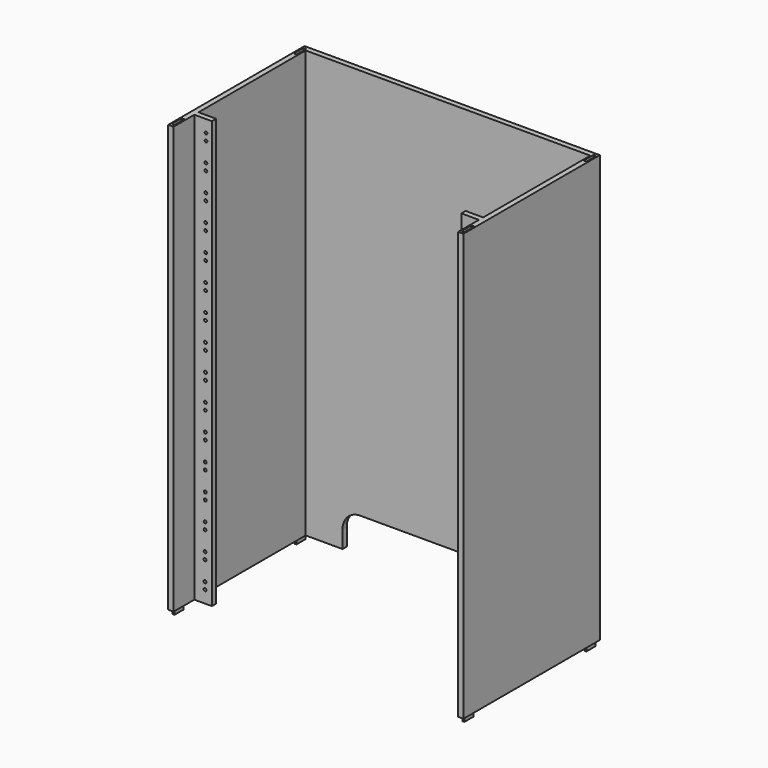
from build123d import *

# Parameters (mm, degrees)
F0_W           = 5
F0_H           = 1.5
F0_W_2         = 0.8
F0_H_2         = 3.5
F0_W_3         = 0.6
F0_H_3         = 3.3
F0_H_4         = 2.7
F0_H_5         = 0.6
F1_DEPTH       = 120
F1_DEPTH_BACK  = 1.5
F3_D           = 0.8
F3_DEPTH       = 2
F3_TIP         = 0.2403442476
F5_D           = 0.8
F5_DEPTH       = 2
F5_TIP         = 0.2403442476
F6_DEPTH       = 2.8
F7_START       = 118.5
F7_DEPTH       = 1.5
F9_DEPTH       = 2
F8_W           = 0.6850839148
F8_H           = 0.2457201043
F8_H_2         = 4.5210258344
F8_TEXT_SIZE   = 11.0822510823
F8_TEXT_SIZE_2 = 3.2900824577
F10_DEPTH      = 0.2


# Not quite as in the source:
# - Text() gives the source's letters only with a copy of the font that has no kerning and outlines rounded to 1/6400 em; it was checked with that copy


with BuildPart() as f1:
    # F0 (on Top) → F1 (new body, two sides)
    with BuildSketch(Plane.XY) as f1_sk:
        with Locations((-38.0453250408, -14.9690947816)):
            Rectangle(F0_W, F0_H)
        Polygon((-42.0453250408, -23.1190947816), (-40.5453250408, -23.1190947816), (-40.5453250408, -15.7190947816), (-40.5453250408, -14.2190947816), (-40.5453250408, 23.8809052184), (-40.8953250408, 23.8809052184), (-40.8953250408, 21.0809052184), (-41.6953250408, 21.0809052184), (-41.6953250408, 23.8809052184), (-42.0453250408, 23.8809052184), align=None)
        with Locations((-41.2953250408, -20.5690947816)):
            Rectangle(F0_W_2, F0_H_2, mode=Mode.SUBTRACT)
        Polygon((-42.0453250408, 25.3809052184), (-42.0453250408, 23.8809052184), (-41.6953250408, 23.8809052184), (-41.6953250408, 24.5809052184), (-40.8953250408, 24.5809052184), (-40.8953250408, 23.8809052184), (-40.5453250408, 23.8809052184), (40.4546749592, 23.8809052184), (40.8046749592, 23.8809052184), (40.8046749592, 24.5809052184), (41.6046749592, 24.5809052184), (41.6046749592, 23.8809052184), (41.9546749592, 23.8809052184), (41.9546749592, 25.3809052184), align=None)
        Polygon((40.8046749592, 23.8809052184), (40.4546749592, 23.8809052184), (40.4546749592, -14.2186603174), (40.4546749592, -15.7186603174), (40.4546749592, -23.1190947816), (41.9546749592, -23.1190947816), (41.9546749592, 23.8809052184), (41.6046749592, 23.8809052184), (41.6046749592, 21.0809052184), (40.8046749592, 21.0809052184), align=None)
        with Locations((41.2046749592, -20.5690947816)):
            Rectangle(F0_W_2, F0_H_2, mode=Mode.SUBTRACT)
        with Locations((37.9546749592, -14.9686603174)):
            Rectangle(F0_W, F0_H)
        with Locations((-41.2953250408, -20.5690947816)):
            Rectangle(F0_W_2, F0_H_2)
        with Locations((-41.2953250408, -20.5690947816)):
            Rectangle(F0_W_3, F0_H_3, mode=Mode.SUBTRACT)
        with Locations((41.2046749592, -20.5690947816)):
            Rectangle(F0_W_2, F0_H_2)
        with Locations((41.2046749592, -20.5690947816)):
            Rectangle(F0_W_3, F0_H_3, mode=Mode.SUBTRACT)
        Polygon((40.9046749592, 23.8809052184), (40.8046749592, 23.8809052184), (40.8046749592, 21.0809052184), (41.6046749592, 21.0809052184), (41.6046749592, 23.8809052184), (41.5046749592, 23.8809052184), (41.5046749592, 21.1809052184), (40.9046749592, 21.1809052184), align=None)
        Polygon((40.8046749592, 24.5809052184), (40.8046749592, 23.8809052184), (40.9046749592, 23.8809052184), (40.9046749592, 24.4809052184), (41.5046749592, 24.4809052184), (41.5046749592, 23.8809052184), (41.6046749592, 23.8809052184), (41.6046749592, 24.5809052184), align=None)
        Polygon((-41.6953250408, 24.5809052184), (-41.6953250408, 23.8809052184), (-41.5953250408, 23.8809052184), (-41.5953250408, 24.4809052184), (-40.9953250408, 24.4809052184), (-40.9953250408, 23.8809052184), (-40.8953250408, 23.8809052184), (-40.8953250408, 24.5809052184), align=None)
        Polygon((-41.5953250408, 23.8809052184), (-41.6953250408, 23.8809052184), (-41.6953250408, 21.0809052184), (-40.8953250408, 21.0809052184), (-40.8953250408, 23.8809052184), (-40.9953250408, 23.8809052184), (-40.9953250408, 21.1809052184), (-41.5953250408, 21.1809052184), align=None)
        with Locations((-41.2953250408, -20.5690947816)):
            Rectangle(F0_W_3, F0_H_3)
        with Locations((-41.2953250408, 22.5309052184)):
            Rectangle(F0_W_3, F0_H_4)
        with Locations((41.2046749592, -20.5690947816)):
            Rectangle(F0_W_3, F0_H_3)
        with Locations((41.2046749592, 22.5309052184)):
            Rectangle(F0_W_3, F0_H_4)
        with Locations((41.2046749592, 24.1809052184)):
            Rectangle(F0_W_3, F0_H_5)
        with Locations((-41.2953250408, 24.1809052184)):
            Rectangle(F0_W_3, F0_H_5)
    extrude(amount=F1_DEPTH)
    extrude(f1_sk.sketch, amount=-F1_DEPTH_BACK)

    # F3
    with Locations(Plane.XZ.offset(15.7190947816)):
        with Locations((-37.4021417661, 48.9999993108), (-37.4021417661, 46.9999994487), (-37.3652911213, 54.4999993108), (-37.3652911213, 56.499999173), (-37.3652911213, 61.999999173), (-37.3652911213, 63.9999990351), (-37.2178886152, 116.4999982081), (-37.2178886152, 114.499998346), (-37.25473926, 108.999998346), (-37.25473926, 106.9999984838), (-37.25473926, 101.4999984838), (-37.25473926, 99.4999986216), (-37.2915899048, 93.9999986216), (-37.2915899048, 91.9999987595), (-37.2915898317, 86.4999987595), (-37.2915898317, 84.4999988973), (-37.3284404765, 78.9999988973), (-37.3284404765, 76.9999988973), (-37.3284404765, 71.4999988973), (-37.3652911213, 69.4999990351), (-37.4021417661, 41.4999994487), (-37.4021417661, 39.4999995865), (-37.4389924109, 33.9999995865), (-37.4389924109, 31.9999997243), (-37.4389923377, 26.4999997243), (-37.4389923377, 24.4999998622), (-37.4758429825, 18.9999998622), (-37.4758429825, 16.9999998622), (-37.4758429825, 11.4999998622), (-37.5126936273, 9.5), (-37.5126936273, 3.9999998622), (-37.5126936273, 2)):
            Hole(F3_D / 2, depth=F3_DEPTH)
            with Locations((0, 0, -(F3_DEPTH + F3_TIP / 2))):  # 118° drill point
                Cone(0, F3_D / 2, F3_TIP, mode=Mode.SUBTRACT)

    # F5
    with Locations(Plane.XZ.offset(15.7186603174)):
        with Locations((37.7800872084, 116.499998536), (37.7800872084, 114.4999986738), (37.7432365636, 108.9999986738), (37.7432365636, 106.9999988116), (37.7432365636, 101.4999988116), (37.7432365636, 99.4999989495), (37.7063859188, 91.9999990873), (37.7063859188, 93.9999989495), (37.7063859919, 86.4999990873), (37.7063859919, 84.4999992251), (37.6695353471, 78.9999992251), (37.6695353471, 76.9999992251), (37.6695353471, 71.4999992251), (37.6326847023, 69.499999363), (37.6326847023, 63.999999363), (37.6326847023, 61.9999995008), (37.6326847023, 56.4999995008), (37.6326847023, 54.4999996386), (37.5958340575, 48.9999996386), (37.5958340575, 46.9999997765), (37.5958340575, 41.4999997765), (37.5958340575, 39.4999999143), (37.5589834127, 33.9999999143), (37.5589834127, 32.0000000522), (37.5589834859, 26.5000000522), (37.5589834859, 24.50000019), (37.5221328411, 19.00000019), (37.5221328411, 17.00000019), (37.5221328411, 11.50000019), (37.4725908041, 9.5000003278), (37.4725908041, 4.00000019), (37.4725908041, 2.0000003278)):
            Hole(F5_D / 2, depth=F5_DEPTH)
            with Locations((0, 0, -(F5_DEPTH + F5_TIP / 2))):  # 118° drill point
                Cone(0, F5_D / 2, F5_TIP, mode=Mode.SUBTRACT)

    # F0 (on Top) → F6 (join)
    with BuildSketch(Plane.XY):
        with Locations((-41.2953250408, 22.5309052184)):
            Rectangle(F0_W_3, F0_H_4)
        with Locations((-41.2953250408, 24.1809052184)):
            Rectangle(F0_W_3, F0_H_5)
        with Locations((-41.2953250408, -20.5690947816)):
            Rectangle(F0_W_3, F0_H_3)
        with Locations((41.2046749592, 22.5309052184)):
            Rectangle(F0_W_3, F0_H_4)
        with Locations((41.2046749592, 24.1809052184)):
            Rectangle(F0_W_3, F0_H_5)
        with Locations((41.2046749592, -20.5690947816)):
            Rectangle(F0_W_3, F0_H_3)
    extrude(amount=-F6_DEPTH)

    # F0 (on Top) → F7 (cut)
    with BuildSketch(Plane.XY.offset(F7_START)):
        with Locations((-41.2953250408, -20.5690947816)):
            Rectangle(F0_W_2, F0_H_2)
        with Locations((-41.2953250408, -20.5690947816)):
            Rectangle(F0_W_3, F0_H_3, mode=Mode.SUBTRACT)
        with Locations((41.2046749592, -20.5690947816)):
            Rectangle(F0_W_2, F0_H_2)
        with Locations((41.2046749592, -20.5690947816)):
            Rectangle(F0_W_3, F0_H_3, mode=Mode.SUBTRACT)
        with Locations((-41.2953250408, -20.5690947816)):
            Rectangle(F0_W_3, F0_H_3)
        with Locations((41.2046749592, -20.5690947816)):
            Rectangle(F0_W_3, F0_H_3)
        with Locations((-41.2953250408, 22.5309052184)):
            Rectangle(F0_W_3, F0_H_4)
        with Locations((41.2046749592, 22.5309052184)):
            Rectangle(F0_W_3, F0_H_4)
        Polygon((-41.5953250408, 23.8809052184), (-41.6953250408, 23.8809052184), (-41.6953250408, 21.0809052184), (-40.8953250408, 21.0809052184), (-40.8953250408, 23.8809052184), (-40.9953250408, 23.8809052184), (-40.9953250408, 21.1809052184), (-41.5953250408, 21.1809052184), align=None)
        Polygon((40.9046749592, 23.8809052184), (40.8046749592, 23.8809052184), (40.8046749592, 21.0809052184), (41.6046749592, 21.0809052184), (41.6046749592, 23.8809052184), (41.5046749592, 23.8809052184), (41.5046749592, 21.1809052184), (40.9046749592, 21.1809052184), align=None)
        with Locations((-41.2953250408, 24.1809052184)):
            Rectangle(F0_W_3, F0_H_5)
        with Locations((41.2046749592, 24.1809052184)):
            Rectangle(F0_W_3, F0_H_5)
        Polygon((40.8046749592, 24.5809052184), (40.8046749592, 23.8809052184), (40.9046749592, 23.8809052184), (40.9046749592, 24.4809052184), (41.5046749592, 24.4809052184), (41.5046749592, 23.8809052184), (41.6046749592, 23.8809052184), (41.6046749592, 24.5809052184), align=None)
        Polygon((-41.6953250408, 24.5809052184), (-41.6953250408, 23.8809052184), (-41.5953250408, 23.8809052184), (-41.5953250408, 24.4809052184), (-40.9953250408, 24.4809052184), (-40.9953250408, 23.8809052184), (-40.8953250408, 23.8809052184), (-40.8953250408, 24.5809052184), align=None)
    extrude(amount=F7_DEPTH, mode=Mode.SUBTRACT)

    # F8 (on face) → F9 (cut)
    with BuildSketch(Plane(origin=(0, 25.3809052184, 0), x_dir=(-1, 0, 0), z_dir=(0, 1, 0))):
        with BuildLine():
            Line((-29.9546749592, 3.5), (-29.9546749592, -1.5))
            Line((-29.9546749592, -1.5), (30.0453250408, -1.5))
            Line((30.0453250408, -1.5), (30.0453250408, 3.5))
            ThreePointArc((30.0453250408, 3.5), (28.5808589467, 7.0355339059), (25.0453250408, 8.5))
            Line((25.0453250408, 8.5), (-24.9546749592, 8.5))
            ThreePointArc((-24.9546749592, 8.5), (-28.4902088651, 7.0355339059), (-29.9546749592, 3.5))
        make_face()
    extrude(amount=-F9_DEPTH, mode=Mode.SUBTRACT)

    # F8 (on face) → F10 (cut)
    with BuildSketch(Plane(origin=(0, 25.3809052184, 0), x_dir=(-1, 0, 0), z_dir=(0, 1, 0))):
        with BuildLine():
            Line((-29.9546749592, 3.5), (-29.9546749592, -1.5))
            Line((-29.9546749592, -1.5), (30.0453250408, -1.5))
            Line((30.0453250408, -1.5), (30.0453250408, 3.5))
            ThreePointArc((30.0453250408, 3.5), (28.5808589467, 7.0355339059), (25.0453250408, 8.5))
            Line((25.0453250408, 8.5), (-24.9546749592, 8.5))
            ThreePointArc((-24.9546749592, 8.5), (-28.4902088651, 7.0355339059), (-29.9546749592, 3.5))
        make_face()
        with Locations((-15.2366672452, 115.9029751797)):
            Rectangle(F8_W, F8_H)
        with BuildLine():
            Line((-14.8941252878, 115.7801151276), (-15.5792092025, 115.7801151276))
            Line((-15.5792092025, 115.7801151276), (-15.5792092025, 109.6066385508))
            Line((-15.5792092025, 109.6066385508), (-15.0881663966, 109.6066385508))
            Line((-15.0881663966, 109.6066385508), (-14.9442855744, 110.1887618772))
            Line((-14.9442855744, 110.1887618772), (-14.8941252878, 110.1887618772))
            add(Edge.make_bspline(
                [(-14.2823017916, 109.6864990071), (-14.6472838773, 109.8495199387), (-14.8941252878, 110.1887618772)],
                knots=[0, 0, 0, 1, 1, 1], degree=2))
            add(Edge.make_bspline(
                [(-13.4751171792, 109.5234780756), (-13.917319706, 109.5234780756), (-14.2823017916, 109.6864990071)],
                knots=[0, 0, 0, 1, 1, 1], degree=2))
            add(Edge.make_bspline(
                [(-12.0950492931, 110.1405816019), (-12.592032133, 109.5234780756), (-13.4751171792, 109.5234780756)],
                knots=[0, 0, 0, 1, 1, 1], degree=2))
            add(Edge.make_bspline(
                [(-11.5980664532, 111.8717714944), (-11.5980664532, 110.7576851282), (-12.0950492931, 110.1405816019)],
                knots=[0, 0, 0, 1, 1, 1], degree=2))
            add(Edge.make_bspline(
                [(-12.0910892704, 113.5930613303), (-11.5980664532, 112.984537853), (-11.5980664532, 111.8717714944)],
                knots=[0, 0, 0, 1, 1, 1], degree=2))
            add(Edge.make_bspline(
                [(-13.4751171792, 114.2015848076), (-12.5841120877, 114.2015848076), (-12.0910892704, 113.5930613303)],
                knots=[0, 0, 0, 1, 1, 1], degree=2))
            add(Edge.make_bspline(
                [(-14.8941252878, 113.5257409456), (-14.4162825572, 114.2015848076), (-13.4751171792, 114.2015848076)],
                knots=[0, 0, 0, 1, 1, 1], degree=2))
            Line((-14.8941252878, 113.5257409456), (-14.9271254763, 113.5257409456))
            add(Edge.make_bspline(
                [(-14.8941252878, 114.4655863162), (-14.8941252878, 113.9415433216), (-14.9271254763, 113.5257409456)],
                knots=[0, 0, 0, 1, 1, 1], degree=2))
            Line((-14.8941252878, 114.4655863162), (-14.8941252878, 115.7801151276))
        make_face()
        with BuildLine():
            add(Edge.make_bspline(
                [(-13.5741177449, 113.628701534), (-14.2750417502, 113.628701534), (-14.584583519, 113.2267592372)],
                knots=[0, 0, 0, 1, 1, 1], degree=2))
            add(Edge.make_bspline(
                [(-12.61777228, 113.1957390599), (-12.9273140489, 113.628701534), (-13.5741177449, 113.628701534)],
                knots=[0, 0, 0, 1, 1, 1], degree=2))
            add(Edge.make_bspline(
                [(-12.3082305112, 111.8796915396), (-12.3082305112, 112.7627765858), (-12.61777228, 113.1957390599)],
                knots=[0, 0, 0, 1, 1, 1], degree=2))
            add(Edge.make_bspline(
                [(-12.61777228, 110.5577039854), (-12.3082305112, 111.0177266141), (-12.3082305112, 111.8796915396)],
                knots=[0, 0, 0, 1, 1, 1], degree=2))
            add(Edge.make_bspline(
                [(-13.5582776544, 110.0976813567), (-12.9273140489, 110.0976813567), (-12.61777228, 110.5577039854)],
                knots=[0, 0, 0, 1, 1, 1], degree=2))
            add(Edge.make_bspline(
                [(-14.5766634737, 110.5082037026), (-14.2592016596, 110.0976813567), (-13.5582776544, 110.0976813567)],
                knots=[0, 0, 0, 1, 1, 1], degree=2))
            add(Edge.make_bspline(
                [(-14.8941252878, 111.8717714944), (-14.8941252878, 110.9187260484), (-14.5766634737, 110.5082037026)],
                knots=[0, 0, 0, 1, 1, 1], degree=2))
            add(Edge.make_bspline(
                [(-14.584583519, 113.2267592372), (-14.8941252878, 112.8248169403), (-14.8941252878, 111.8717714944)],
                knots=[0, 0, 0, 1, 1, 1], degree=2))
        make_face(mode=Mode.SUBTRACT)
        with BuildLine():
            add(Edge.make_bspline(
                [(12.9642700032, 115.7801151276), (13.0358619878, 115.8067139798), (13.1217148027, 115.8067139798)],
                knots=[0.5072754569, 0.5072754569, 0.5072754569, 1, 1, 1], degree=2))
            Line((12.9642700032, 115.7801151276), (13.272005287, 115.7801151276))
            add(Edge.make_bspline(
                [(13.1217148027, 115.8067139798), (13.2022899881, 115.8067139798), (13.272005287, 115.7801151276)],
                knots=[0, 0, 0, 0.488331666, 0.488331666, 0.488331666], degree=2))
        make_face()
        with BuildLine():
            Line((13.272005287, 115.7801151276), (12.9642700032, 115.7801151276))
            add(Edge.make_bspline(
                [(12.8319731471, 115.6971533537), (12.8905637971, 115.7527307703), (12.9642700032, 115.7801151276)],
                knots=[0, 0, 0, 0.5072754569, 0.5072754569, 0.5072754569], degree=2))
            add(Edge.make_bspline(
                [(12.7164724871, 115.352631385), (12.7164724871, 115.5875927276), (12.8319731471, 115.6971533537)],
                knots=[0, 0, 0, 1, 1, 1], degree=2))
            add(Edge.make_bspline(
                [(12.8319731471, 115.0081094163), (12.7164724871, 115.121630065), (12.7164724871, 115.352631385)],
                knots=[0, 0, 0, 1, 1, 1], degree=2))
            add(Edge.make_bspline(
                [(13.1217148027, 114.8945887676), (12.9474738071, 114.8945887676), (12.8319731471, 115.0081094163)],
                knots=[0, 0, 0, 1, 1, 1], degree=2))
            add(Edge.make_bspline(
                [(13.4061764282, 115.0081094163), (13.2867157456, 114.8945887676), (13.1217148027, 114.8945887676)],
                knots=[0, 0, 0, 1, 1, 1], degree=2))
            add(Edge.make_bspline(
                [(13.5256371109, 115.352631385), (13.5256371109, 115.121630065), (13.4061764282, 115.0081094163)],
                knots=[0, 0, 0, 1, 1, 1], degree=2))
            add(Edge.make_bspline(
                [(13.4061764282, 115.6951733424), (13.5256371109, 115.583632705), (13.5256371109, 115.352631385)],
                knots=[0, 0, 0, 1, 1, 1], degree=2))
            add(Edge.make_bspline(
                [(13.272005287, 115.7801151276), (13.3450521798, 115.7522451545), (13.4061764282, 115.6951733424)],
                knots=[0.488331666, 0.488331666, 0.488331666, 1, 1, 1], degree=2))
        make_face()
        Polygon((-7.0652619935, 71.9479341183), (-7.0647909463, 71.9476771835), (-7.1052153615, 71.9464781542), (-7.3177861214, 71.8939778014), (-7.5480425629, 71.7664524744), (-7.5972884077, 71.7274412008), (-7.6848603666, 71.7613566001), (-7.9564404954, 71.8394219698), (-8.306557041, 71.8754356702), (-8.6448117614, 71.8054637481), (-8.8975928241, 71.6626079755), (-8.9675219238, 71.5991450694), (-9.0688398968, 71.6124200362), (-9.3769047732, 71.6175159106), (-9.6587194732, 71.5608617778), (-9.8489754419, 71.4504654404), (-9.9537620353, 71.3463640066), (-9.9839604438, 71.3078237802), (-10.0057999054, 71.3082948274), (-10.071314008, 71.3139045715), (-10.2165164521, 71.3222121314), (-10.4049353368, 71.3222121314), (-10.6212316519, 71.3034558879), (-10.8507729581, 71.2548523802), (-11.0784514867, 71.1658672796), (-11.289403557, 71.0260519027), (-11.4313557754, 70.8796846874), (-11.4685299649, 70.8241439389), (-11.5584357486, 70.8348495573), (-11.8323539844, 70.832023274), (-12.1283386409, 70.7688601252), (-12.3564796522, 70.6449747086), (-12.5170168242, 70.471929092), (-12.6099501568, 70.2600434917), (-12.6355066091, 70.0204945734), (-12.5936904635, 69.7640307779), (-12.5186483604, 69.5635359557), (-12.4847243967, 69.5012720788), (-12.525148812, 69.4390082019), (-12.6371295809, 69.2457075552), (-12.723095697, 68.9623084238), (-12.6736057641, 68.6219125797), (-12.4956441275, 68.2917513068), (-12.4192102941, 68.1951009835), (-12.4508047152, 68.1326229942), (-12.4988943533, 67.9216366659), (-12.4677666971, 67.6319426308), (-12.3239559834, 67.3213512284), (-12.1360038637, 67.0637312261), (-12.0651455163, 66.9851519867), (-12.0839659936, 66.9007917134), (-12.0893059561, 66.6364485827), (-12.0040421285, 66.3362630415), (-11.8242219966, 66.0783861044), (-11.6344113816, 65.9048266182), (-11.5647135232, 65.8560518205), (-11.5767894608, 65.7443279864), (-11.4943176586, 65.3955817599), (-11.2520024084, 65.0398982927), (-10.9564802346, 64.7859610232), (-10.7794478457, 64.6663150314), (-10.7269432106, 64.6307295557), (-10.7120752477, 64.5563897412), (-10.6416793831, 64.3380807699), (-10.4725434584, 64.0673999131), (-10.1681955727, 63.8322617096), (-9.8036735469, 63.6795995905), (-9.6773044268, 63.6466691082), (-9.6563642371, 63.5520742636), (-9.5183902266, 63.2848620272), (-9.2625687682, 63.0593160578), (-8.9440552082, 62.9220272069), (-8.6840799699, 62.8476445699), (-8.5969790582, 62.8241778543), (-8.7409910375, 62.740545563), (-9.1627067593, 62.4721771198), (-9.6947331736, 62.0767972193), (-10.1802800748, 61.6214658556), (-10.605896924, 61.0889683941), (-10.9590367363, 60.4630322948), (-11.2264459561, 59.7267855031), (-11.3951108336, 58.8635272541), (-11.4527327543, 58.1077534143), (-11.4518035066, 57.8558716236), (-11.6776192576, 57.4530406127), (-11.7631186088, 57.4012254194), (-12.0061361475, 57.2244114252), (-12.3246497075, 56.944480914), (-12.6276058627, 56.6173600368), (-12.9094205627, 56.2479305555), (-13.1640472741, 55.8404747175), (-13.3859233575, 55.3992747701), (-13.5694604801, 54.928998363), (-13.7088561967, 54.4339277436), (-13.79830378, 53.9183879817), (-13.8322234615, 53.3873036619), (-13.8048085138, 52.8445716292), (-13.7104834508, 52.2946454209), (-13.5434372628, 51.7424496214), (-13.2978675046, 51.1920523659), (-12.9681986902, 50.647950014), (-12.6610630615, 50.2411365131), (-12.5486198098, 50.1142963458), (-12.5200400908, 49.9588507659), (-12.4085218046, 49.4964965165), (-12.2400881685, 48.941945481), (-12.0565467636, 48.4213098448), (-11.9162260815, 48.0344944391), (-11.8711468634, 47.904870811), (-11.8390899595, 47.6553014338), (-11.6485856204, 46.9184123049), (-11.2817383342, 46.0685574902), (-10.814990499, 45.3508956521), (-10.2917983611, 44.7621722825), (-9.7565260033, 44.2979766667), (-9.2528480666, 43.9546132252), (-8.8246661513, 43.7280951856), (-8.5953518042, 43.6342326054), (-8.5158732928, 43.6142516391), (-8.3430417887, 43.4827566689), (-7.8140129476, 43.1008101784), (-7.0631208698, 42.6159398723), (-6.236304546, 42.1747570539), (-5.5437366775, 41.8755178894), (-5.30697122, 41.7923480808), (-5.0897756329, 41.5683865429), (-4.3565692368, 40.9747899758), (-3.376362812, 40.4260328211), (-2.3752590199, 40.118199186), (-1.6153314001, 40.0220156277), (-1.3620792902, 40.0220156277), (-1.3472198918, 40.0220156277), (-1.3072237013, 40.0220156277), (-1.3021278269, 40.0220156277), (-1.0491326518, 40.0220156277), (-0.289205032, 40.1179679447), (0.71189876, 40.4260328211), (1.6921051849, 40.9747899758), (2.425311581, 41.5683865429), (2.6427641029, 41.7923480808), (2.8792298031, 41.8755178894), (3.5718404941, 42.1747570539), (4.3984427055, 42.6159398723), (5.1495488956, 43.1008101784), (5.6785777367, 43.4827566689), (5.8516661758, 43.6142516391), (5.9308877523, 43.6339970818), (6.1602020994, 43.7280951856), (6.5881699024, 43.9546132252), (7.091847839, 44.2979766667), (7.6273856961, 44.7621722825), (8.1502909235, 45.3508956521), (8.61727, 46.0685574902), (8.9841301329, 46.9184123049), (9.1746473188, 47.6553014338), (9.206935464, 47.904870811), (9.2517705941, 48.0344944391), (9.3920570182, 48.4213098448), (9.5755941408, 48.941945481), (9.7440577527, 49.4964965165), (9.8555674744, 49.9588507659), (9.8844298217, 50.1142963458), (9.9965818806, 50.2411365131), (10.3037903075, 50.647950014), (10.6333948882, 51.1920523659), (10.8789817753, 51.7426637338), (11.0460322456, 52.2949023557), (11.1403701553, 52.844828564), (11.1677765385, 53.3875177743), (11.1338611393, 53.918859029), (11.0444049916, 54.4341846785), (10.9050178394, 54.9292552978), (10.7214807168, 55.3997029948), (10.4995746576, 55.8409029422), (10.2446952937, 56.2484016027), (9.9631375286, 56.617831084), (9.6601685266, 56.9449519613), (9.3414408542, 57.2248824724), (9.0984233155, 57.4016964666), (9.0131637702, 57.4535116599), (8.7871467536, 57.8563426708), (8.7877890907, 58.1081816391), (8.7301500409, 58.8637413665), (8.5615579617, 59.727042438), (8.2940887904, 60.4632892297), (7.9409746716, 61.089225329), (7.5153621047, 61.621679968), (7.0297980745, 62.0770541542), (6.4977288377, 62.4726909895), (6.0760559384, 62.7410166102), (5.9323008939, 62.8246489015), (6.0191448707, 62.8479015047), (6.2791629315, 62.9222413192), (6.5976764915, 63.0595301702), (6.8534551274, 63.2851189621), (6.9914719604, 63.5525024884), (7.0126262625, 63.6470973329), (7.1387812702, 63.6798565254), (7.5032861671, 63.8326899343), (7.8078824231, 64.0676140255), (7.9769883721, 64.3384661722), (8.0471315841, 64.5568607884), (8.0622479174, 64.6312006029), (8.1145341579, 64.6667860786), (8.2917763768, 64.7864320704), (8.587080156, 65.0403693399), (8.8293697127, 65.3960956296), (8.9118457972, 65.7447990336), (8.9000267944, 65.8565228677), (8.9694848469, 65.9052976654), (9.1595309856, 66.0788571516), (9.3393853754, 66.3367340887), (9.4243879859, 66.6369196299), (9.4190779992, 66.9015196955), (9.4004502231, 66.985623034), (9.4711073048, 67.0641166284), (9.6590551422, 67.3217794532), (9.8028530092, 67.632413678), (9.8339849476, 67.9221077131), (9.7858524871, 68.1330940414), (9.7545064363, 68.1956148532), (9.830944552, 68.2920082416), (10.008914753, 68.6221695145), (10.0584175327, 68.9624797136), (9.972215893, 69.2459216676), (9.8601923016, 69.4392223143), (9.8200676437, 69.5014861911), (9.853726108, 69.5637928905), (9.9287939046, 69.7642877127), (9.9703745266, 70.0207086858), (9.9447666873, 70.2603004266), (9.8518847417, 70.4721432044), (9.6913432875, 70.6452316434), (9.4631851472, 70.7688601252), (9.1671962084, 70.8322802089), (8.8933036661, 70.8348495573), (8.8033764711, 70.8241439389), (8.7662065639, 70.8796846874), (8.6242500633, 71.0260519027), (8.413263735, 71.1658672796), (8.1856194643, 71.2548523802), (7.9563479397, 71.3034558879), (7.7397946898, 71.3224690663), (7.5515899175, 71.3222121314), (7.4061647965, 71.3140758614), (7.3406464117, 71.3085517623), (7.3190638849, 71.3080807151), (7.288617106, 71.3466209415), (7.1837876902, 71.4506795528), (6.9935274392, 71.5610758902), (6.7119696741, 71.6177728455), (6.4039047977, 71.6126341486), (6.3028437595, 71.5994020042), (6.232657725, 71.6628649104), (5.9798766623, 71.8057206829), (5.6416647643, 71.8756497826), (5.2915053962, 71.8395932597), (5.01996809, 71.7613566001), (4.932567421, 71.7276981357), (4.8466227161, 71.7954861117), (4.5348322845, 71.9305053715), (4.1865999277, 71.9251525623), (3.8645749248, 71.8092321258), (3.6271671302, 71.7060299639), (3.5456331401, 71.6802936572), (3.4419599311, 71.714166234), (3.1139397819, 71.7608855529), (2.8158525419, 71.7074431056), (2.5840116689, 71.5880112262), (2.4118225018, 71.4923458198), (2.3512287014, 71.4697783761), (2.2348372176, 71.4944012985), (1.8716598175, 71.5020665213), (1.5278381755, 71.3896147052), (1.2580994131, 71.1782001521), (1.0652269912, 70.9791184715), (1.0004794109, 70.9133431518), (0.5780785295, 70.9217363566), (0.4726067765, 70.8596865921), (0.1761467905, 70.6394506094), (-0.1741838675, 70.3074479702), (-0.4757825503, 69.9422150913), (-0.7306190918, 69.5593821757), (-0.9413484853, 69.175093296), (-1.1102403219, 68.8052355899), (-1.2400780624, 68.4657818402), (-1.3121054633, 68.2467020644), (-1.333045653, 68.1728332971), (-1.3541571325, 68.2467020644), (-1.4261845334, 68.4657818402), (-1.5558509841, 68.8052355899), (-1.7247428207, 69.175093296), (-1.9352581018, 69.5593821757), (-2.1898805309, 69.9422150913), (-2.4909225216, 70.3074479702), (-2.8410818897, 70.6394506094), (-3.1375418757, 70.8596865921), (-3.2427566938, 70.9217363566), (-3.6651575752, 70.9133431518), (-3.7301620904, 70.9791184715), (-3.9232914471, 71.1782001521), (-4.1932443218, 71.3896147052), (-4.5370659638, 71.5020665213), (-4.900157719, 71.4944012985), (-5.0163350904, 71.4697783761), (-5.0772286481, 71.4923458198), (-5.2493321703, 71.5880112262), (-5.4810017534, 71.7074431056), (-5.7790889934, 71.7608855529), (-6.1073660774, 71.714166234), (-6.2106967067, 71.6802936572), (-6.2644389113, 71.6972085343), (-6.4212548103, 71.7615707124), (-6.6294148553, 71.8514979074), (-6.8419856152, 71.9227973262), (-7.009721245, 71.9497754847), align=None)
        Polygon((-10.9989986688, 56.6926419457), (-10.8772586581, 56.7620999982), (-10.8138300099, 56.7793146327), (-10.6038071873, 56.7585885554), (-10.3900673739, 56.5996743552), (-10.2325534686, 56.3076679064), (-10.1273043925, 55.9052651203), (-10.0708515253, 55.4145623932), (-10.0599317945, 54.8584269262), (-10.090596968, 54.2592548731), (-10.1593698609, 53.6391854527), (-10.2627561593, 53.0211715111), (-10.3970388726, 52.4270953323), (-10.55850101, 51.8799954072), (-10.7439009103, 51.4018824874), (-10.9492774945, 51.0152811941), (-11.171380537, 50.742758971), (-11.4062618057, 50.6067976167), (-11.5974727157, 50.606369392), (-11.6504398335, 50.6298361076), (-11.7199064505, 50.6858479033), (-11.9111087959, 50.8746950127), (-12.1452963405, 51.1660591243), (-12.3499749185, 51.4982758759), (-12.521894304, 51.8651360088), (-12.6582710362, 52.2603017969), (-12.7553838423, 52.6782919635), (-12.8102137377, 53.1126831375), (-12.8197417381, 53.5573945278), (-12.7804778119, 54.0064738103), (-12.6896427805, 54.4539258389), (-12.5437337656, 54.8934985322), (-12.3395176704, 55.319368034), (-12.0739712282, 55.7249825057), (-11.7440668902, 56.1048606706), (-11.3460919478, 56.4526219802), align=None, mode=Mode.SUBTRACT)
        Polygon((-6.7392545006, 48.7261202132), (-6.6294148553, 48.5985948862), (-6.5301951836, 48.4789488945), (-6.268121644, 48.0900351876), (-5.9688781972, 47.5219950729), (-5.7405059445, 46.9235510018), (-5.5925114751, 46.3241220138), (-5.534015976, 45.7530415034), (-5.5734982968, 45.2393859304), (-5.7207647841, 44.8125743342), (-5.904772954, 44.5612064131), (-5.9842086428, 44.501725997), (-6.0667275498, 44.4520091049), (-6.3431466181, 44.351419114), (-6.7915407411, 44.2793917131), (-7.3084508221, 44.2996039207), (-7.8739644109, 44.4250737689), (-8.4673126076, 44.6690334021), (-9.0681119147, 45.0444580297), (-9.6558931899, 45.565093666), (-10.0852570055, 46.0645750002), (-10.2100160006, 46.2437442305), (-10.2964403172, 46.3982477159), (-10.518547642, 46.882355782), (-10.7322831731, 47.5091911532), (-10.8572776918, 48.1093053008), (-10.9000230852, 48.6680529387), (-10.8665701687, 49.1708316034), (-10.7631838702, 49.602739074), (-10.5961376822, 49.9493441768), (-10.4367695638, 50.1458565089), (-10.3714824203, 50.1953592886), (-10.2806431066, 50.2509000371), (-9.9718759417, 50.3587270261), (-9.531622371, 50.3979952346), (-9.0613887864, 50.322927438), (-8.5716281537, 50.1444861898), (-8.0730889139, 49.8724350138), (-7.5759199933, 49.5172225938), (-7.0912552351, 49.0892976133), align=None, mode=Mode.SUBTRACT)
        Polygon((-1.3855888283, 44.4083301817), (-1.2421763636, 44.4046474489), (-1.1011619574, 44.4108995301), (-0.6767484198, 44.4013929409), (-0.093335037, 44.3472225116), (0.4795868398, 44.2468894555), (1.0127694608, 44.105159914), (1.4778643486, 43.9276607602), (1.8460948006, 43.7187984266), (2.088898227, 43.4836859165), (2.1767271207, 43.2915500412), (2.1771981679, 43.2271964276), (2.1795105815, 43.1547065439), (2.1042286726, 42.9337682727), (1.8828364831, 42.5878354828), (1.5343471915, 42.2182004536), (1.0810713065, 41.8534471864), (0.5448482898, 41.5223823593), (-0.0517544149, 41.2535814091), (-0.6871542809, 41.075851014), (-1.1764438663, 41.0147519084), (-1.3390836218, 41.0175353692), (-1.506134092, 41.0103326291), (-2.0102402534, 41.059822562), (-2.6577588794, 41.2240767247), (-3.2604423754, 41.479170201), (-3.7982498237, 41.7944335353), (-4.2505836142, 42.1385121121), (-4.5965463799, 42.48049667), (-4.8155833333, 42.7892595527), (-4.8899231478, 42.9734989639), (-4.8873966218, 43.0336688218), (-4.8899231478, 43.1047584105), (-4.7981545865, 43.3210547256), (-4.5330834738, 43.5863699264), (-4.1281541617, 43.8242744618), (-3.6186523686, 44.0291928456), (-3.0396925231, 44.1952883746), (-2.4270313907, 44.3170326676), (-1.8162972696, 44.3885890213), align=None, mode=Mode.SUBTRACT)
        Polygon((2.3732822754, 48.9747474959), (2.372340181, 48.8099666168), (2.3732822754, 48.6455283175), (2.3051945421, 48.15135697), (2.1014452118, 47.5234082145), (1.7690143478, 46.9441914341), (1.440480329, 46.5471842797), (1.3156956404, 46.4311781982), (1.1888982955, 46.3136733302), (0.7618725869, 46.0107043281), (0.1355082629, 45.7010121977), (-0.5442985084, 45.5100239647), (-1.079793543, 45.4445055798), (-1.2582347913, 45.4445055798), (-1.4368901519, 45.4445055798), (-1.972428009, 45.5100239647), (-2.6521491354, 45.7010121977), (-3.2785562818, 46.0107043281), (-3.7052822331, 46.3136733302), (-3.8321652229, 46.4311781982), (-3.9571640239, 46.5471842797), (-4.2856552203, 46.9441914341), (-4.6181289067, 47.5234082145), (-4.821878237, 48.15135697), (-4.8897518579, 48.6455283175), (-4.8888097635, 48.8099666168), (-4.8897518579, 48.9747474959), (-4.821878237, 49.4686619085), (-4.6181289067, 50.0966106641), (-4.2856552203, 50.6758702669), (-3.9571640239, 51.0728345989), (-3.8321652229, 51.1885837455), (-3.7052822331, 51.3063455484), (-3.2785562818, 51.6093145504), (-2.6521491354, 51.9190066808), (-1.972428009, 52.1099949139), (-1.4368901519, 52.1752991864), (-1.2582347913, 52.1752991864), (-1.079793543, 52.1752991864), (-0.5442985084, 52.1099949139), (0.1355082629, 51.9190066808), (0.7618725869, 51.6093145504), (1.1886413607, 51.3063455484), (1.3156956404, 51.1885837455), (1.440480329, 51.0728345989), (1.7690143478, 50.6758702669), (2.1014452118, 50.0966106641), (2.3051945421, 49.4686619085), align=None, mode=Mode.SUBTRACT)
        Polygon((-3.4962229161, 58.4634368816), (-3.3589340651, 58.3732527518), (-3.221902149, 58.2836253142), (-2.8531150048, 57.9485822793), (-2.4651862148, 57.4270045486), (-2.1980168009, 56.8283035427), (-2.0534909519, 56.1726486466), (-2.0342208387, 55.4805946478), (-2.1429470996, 54.7715401269), (-2.3818108584, 54.0659542264), (-2.6466250362, 53.5450616553), (-2.7532958184, 53.3835781067), (-2.8601378905, 53.2221373805), (-3.2355625182, 52.7739573699), (-3.7917836301, 52.2763602246), (-4.4027746861, 51.8962251248), (-5.048837348, 51.6397613293), (-5.7105302129, 51.5126642271), (-6.3684975226, 51.5201153376), (-7.003212229, 51.6685808542), (-7.458115368, 51.8729725215), (-7.5951901065, 51.9628997165), (-7.7324789575, 52.0528269114), (-8.1012232792, 52.3878699463), (-8.4891520692, 52.9094048545), (-8.7563214831, 53.5081486829), (-8.9008473322, 54.1637607565), (-8.9201602678, 54.8558575778), (-8.8113911844, 55.5649120987), (-8.5725702481, 56.2704979992), (-8.3074991354, 56.7913905703), (-8.2008711757, 56.9526171841), (-8.0942003935, 57.1142720226), (-7.7187757659, 57.5624948557), (-7.1623405415, 58.060092001), (-6.551563598, 58.4401414558), (-5.905500936, 58.6966908963), (-5.2438080711, 58.8237879985), (-4.5855838266, 58.816336888), (-3.9511260551, 58.6678713714), align=None, mode=Mode.SUBTRACT)
        Polygon((3.8287753368, 48.8683336486), (3.937073373, 48.9951738159), (3.937073373, 48.9954307508), (4.0546210635, 49.1283088869), (4.422166356, 49.5139252633), (4.9100427998, 49.9711836384), (5.3942365108, 50.3536311517), (5.8688379878, 50.6470079196), (6.328194664, 50.8377392178), (6.7660972809, 50.9116079851), (7.1768504494, 50.8551679647), (7.4712549567, 50.7187783857), (7.5546303131, 50.6542020952), (7.622675224, 50.5864141192), (7.7813324893, 50.3356885352), (7.9686379897, 49.8826695851), (8.1017302382, 49.32743339), (8.1663493511, 48.7022252728), (8.1479785099, 48.0391620887), (8.0318011385, 47.3707460955), (7.8036429982, 46.728794391), (7.5530030591, 46.2792868837), (7.4489444479, 46.1454666531), (7.3125548689, 45.9563197864), (6.8439485383, 45.4315303702), (6.2094479442, 44.8953073535), (5.5673249499, 44.5207819978), (4.9392905494, 44.2919386979), (4.3473554943, 44.1922908014), (3.8134877136, 44.2055229458), (3.3595266691, 44.3156623484), (3.0858054166, 44.4459711361), (3.0075259346, 44.5059225994), (2.9304026593, 44.5786351599), (2.765878715, 44.8669588759), (2.6488020717, 45.3485832385), (2.6450765165, 45.9191498792), (2.7435682062, 46.5469273448), (2.9329720077, 47.2002270049), (3.2024538352, 47.8472317612), (3.5407513781, 48.4561673384), align=None, mode=Mode.SUBTRACT)
        Polygon((0.5641612255, 58.4620665624), (0.7014500764, 58.551694), (0.838524815, 58.641621195), (1.2932138416, 58.8463126197), (1.9278857256, 58.9947781363), (2.5858530352, 59.0021864242), (3.2477600125, 58.8750893221), (3.8936085621, 58.6185827041), (4.5046424405, 58.2385332493), (5.06082073, 57.7408932815), (5.4362881801, 57.2927132708), (5.5431730746, 57.1310584323), (5.6498010344, 56.9697889961), (5.9146580347, 56.448896425), (6.1534361485, 55.7433533469), (6.2621624094, 55.034298826), (6.2431492311, 54.3421591823), (6.0986233821, 53.6865899312), (5.8311970333, 53.0878461027), (5.4432254208, 52.5662683721), (5.074566744, 52.2312681597), (4.937449183, 52.1413409647), (4.8001175096, 52.0514137698), (4.3455141279, 51.8469792799), (3.7107994215, 51.6985137633), (3.0527892894, 51.6911054754), (2.390967957, 51.8182025776), (1.7450337625, 52.074666373), (1.1340427066, 52.4547586503), (0.5776074823, 52.9523986182), (0.2021828546, 53.4005358063), (0.0955548949, 53.5620193549), (-0.0113299997, 53.7235029036), (-0.276187, 54.2443954746), (-0.5150079363, 54.9499385527), (-0.6235200849, 55.659035896), (-0.604464084, 56.3510898948), (-0.459938235, 57.0067447909), (-0.1925547087, 57.6054029744), (0.1954169038, 58.1270235275), align=None, mode=Mode.SUBTRACT)
        Polygon((7.8282659206, 56.8685138456), (7.8919857616, 56.8513420336), (8.0134731197, 56.7818411586), (8.3605920922, 56.5418211931), (8.7582844062, 56.1940598835), (9.0884456791, 55.8141817186), (9.353987839, 55.4083103121), (9.5579512816, 54.9827405676), (9.7038902723, 54.5429109394), (9.794973674, 54.0957158457), (9.8339849476, 53.6463796283), (9.8244783585, 53.201668238), (9.7696227695, 52.7672342415), (9.672501399, 52.3492440749), (9.53611182, 51.9538641745), (9.3642224102, 51.5870040416), (9.1595309856, 51.2550442248), (8.9253776989, 50.9634660009), (8.734132531, 50.7748330039), (8.6649314134, 50.7187783857), (8.6117030785, 50.6953544925), (8.4204579106, 50.6958255397), (8.1856194643, 50.8317440715), (7.9635421153, 51.1042662947), (7.758165531, 51.4906106531), (7.572787042, 51.9687235729), (7.4113034934, 52.5160804328), (7.2770122156, 53.1098996767), (7.1736387639, 53.7281277307), (7.1048230485, 54.3482399736), (7.0742049798, 54.9474120267), (7.0850818881, 55.5035474937), (7.141564731, 55.9942073983), (7.2467795491, 56.3968671193), (7.4044947201, 56.6886594557), (7.6182645092, 56.8478305907), align=None, mode=Mode.SUBTRACT)
        Polygon((-5.6232151888, 62.310950506), (-5.370605416, 62.2682564996), (-5.3392593652, 62.2631178028), (-5.2561409436, 62.1795283339), (-5.2870159472, 61.9889683256), (-5.4445598282, 61.7137054641), (-5.7098878758, 61.370055112), (-6.0636871542, 60.9753175487), (-6.4876724671, 60.546022249), (-6.9625308789, 60.0989984452), (-7.469506146, 59.6506043223), (-7.9894566226, 59.2180545146), (-8.5040542901, 58.817964142), (-8.9937721003, 58.4671624368), (-9.440067922, 58.1823501637), (-9.8238857545, 57.9799283301), (-10.1263751448, 57.8772828604), (-10.3287284624, 57.8904721824), (-10.4088878511, 57.9989843309), (-10.4116755942, 58.0368393978), (-10.4200388233, 58.3044798589), (-10.3371002561, 59.1106985728), (-10.0580732992, 60.0467122047), (-9.5971407559, 60.8361873314), (-8.9777564951, 61.469745831), (-8.2224537025, 61.9388232088), (-7.354270869, 62.2342982779), (-6.3959039058, 62.3470070289), align=None, mode=Mode.SUBTRACT)
        Polygon((-1.4994109636, 62.9812506881), (-1.344436431, 62.9770969081), (-1.2024371079, 62.9786813397), (-0.7757111567, 62.9322189556), (-0.1992778371, 62.794416235), (0.3585705289, 62.5781627424), (0.8724402143, 62.2972901368), (1.3161666876, 61.9660154797), (1.6644418669, 61.5982132523), (1.8909299307, 61.2085715634), (1.9711364241, 60.9100560987), (1.9706225544, 60.8106223145), (1.9699373948, 60.7253199468), (1.9093007719, 60.4695841333), (1.7345850789, 60.1522267801), (1.4530273138, 59.8654874957), (1.0710508477, 59.6162178758), (0.5950362291, 59.4115264511), (0.0314496516, 59.2581791725), (-0.613499626, 59.1634558605), (-1.1534481979, 59.1325380344), (-1.333045653, 59.1336942412), (-1.5100737596, 59.1357925424), (-2.0406870322, 59.1831970209), (-2.6800693883, 59.306311633), (-3.2427566938, 59.4926322165), (-3.7208696135, 59.7311962179), (-4.1065716349, 60.0109554391), (-4.3914267305, 60.3213327291), (-4.5675127427, 60.6514511795), (-4.6271644487, 60.9056453839), (-4.6267790464, 60.9901769471), (-4.6265221116, 61.0657157909), (-4.5532956814, 61.2915615176), (-4.3474480499, 61.6212089208), (-4.0277782831, 61.9578363872), (-3.611458193, 62.2796044552), (-3.1173296681, 62.5642026159), (-2.5627786326, 62.7897914078), (-1.9656192357, 62.934788304), align=None, mode=Mode.SUBTRACT)
        Polygon((-8.9041018402, 68.8375237352), (-9.3392638187, 68.9857323169), (-9.0681119147, 68.8460882299), (-8.2612508637, 68.4137525346), (-7.2966318193, 67.8680229287), (-6.4400538762, 67.3480724521), (-5.6856503556, 66.8518028034), (-5.0282397381, 66.3785716456), (-4.4617840549, 65.9268801922), (-3.9813158991, 65.4952724789), (-3.6769765779, 65.1895200161), (-3.5810542366, 65.0824210092), (-3.623748243, 64.9114308714), (-3.8570450802, 64.4247106344), (-4.2847559483, 63.9238161585), (-4.8204650953, 63.5592684392), (-5.4210502901, 63.3106839789), (-6.0425328521, 63.1575936351), (-6.6414907929, 63.0792713306), (-7.1744593016, 63.0558474374), (-7.4918166548, 63.0602153298), (-7.5972884077, 63.066296121), (-7.5621739792, 63.0827827734), (-7.4596997995, 63.1378524747), (-7.3407389673, 63.2196433996), (-7.2471290396, 63.3153088061), (-7.1962987632, 63.3991980322), (-7.1858072572, 63.4291737639), (-7.2413480057, 63.4686560847), (-7.4629543075, 63.5081384055), (-7.8858262361, 63.5423535621), (-8.3739167923, 63.6069298525), (-8.739406606, 63.7153991786), (-8.8471907725, 63.7760358015), (-8.8100208653, 63.7839151367), (-8.6991963031, 63.8127346615), (-8.5846461857, 63.8603532524), (-8.4926635121, 63.9305392869), (-8.4294575408, 64.0067204678), (-8.4118146816, 64.034126851), (-8.5163443401, 64.0673999131), (-8.8304471853, 64.1645212837), (-9.2379458458, 64.3010821525), (-9.6073753271, 64.4595253055), (-9.8429417554, 64.5977990734), (-9.9117060838, 64.6551811882), (-9.8766259132, 64.6549670759), (-9.7711284668, 64.6502994262), (-9.6271164875, 64.6544532062), (-9.4723560673, 64.6914090011), (-9.3390068839, 64.7564563387), (-9.2988394035, 64.7841196568), (-9.42289611, 64.8510511833), (-10.0485452987, 65.1748747301), (-10.6316889, 65.5691412462), (-10.7343771921, 65.6711443787), (-10.6865187954, 65.6723005855), (-10.5420100754, 65.6757692059), (-10.3621856612, 65.6866889367), (-10.2153559631, 65.7140953199), (-10.137992882, 65.7486958788), (-10.1214976651, 65.767965992), (-10.235105688, 65.8384089613), (-10.7494806786, 66.2131484294), (-11.195545259, 66.6180777415), (-11.2747668355, 66.7033372868), (-11.217149197, 66.6966141584), (-11.0424377862, 66.6852233804), (-10.8744666328, 66.6922462661), (-10.7573771428, 66.7187105549), (-10.6960425136, 66.74701621), (-10.6779200427, 66.7597773072), (-10.7429716626, 66.8262377865), (-10.9474189992, 67.0160698128), (-11.2208661877, 67.2697501475), (-11.4689924476, 67.5385896379), (-11.6234916507, 67.7604100521), (-11.661822047, 67.840573723), (-11.6141948917, 67.8243440055), (-11.4671382345, 67.7843906374), (-11.2852240836, 67.759767715), (-11.120036391, 67.777667509), (-11.0075931393, 67.8248150527), (-10.9762299595, 67.8487528155), (-10.9996923929, 67.9014672807), (-11.1263098834, 68.0346023517), (-11.3639831774, 68.2332558076), (-11.6337176575, 68.4975989383), (-11.8318872194, 68.778942591), (-11.879518657, 68.8809457236), (-11.8272452632, 68.8760639616), (-11.6701852762, 68.8609476283), (-11.4782892066, 68.8479724188), (-11.3277382356, 68.8514410391), (-11.2566443646, 68.8665573724), (-11.242474408, 68.8809457236), (-11.2647763524, 68.9720291253), (-11.356082431, 69.2389844269), (-11.4954781476, 69.5323611947), (-11.6513690812, 69.7844999204), (-11.7735715746, 69.959900773), (-11.8146939962, 70.0177539351), (-11.6927227441, 70.0195953014), (-11.3265777465, 70.0221646499), (-10.8405469513, 70.0263184298), (-10.4746374774, 70.0386084798), (-10.347086457, 70.0662717979), (-10.7178776929, 70.4452078684), (-10.6119434573, 70.4738132808), (-10.2787846113, 70.5058873137), (-9.8510694609, 70.4747125528), (-9.4517156349, 70.3887678479), (-9.1852313805, 70.3116017502), (-9.0969314396, 70.2839812546), (-9.0699961036, 70.3053924915), (-9.0188660699, 70.4068817543), (-9.0553508176, 70.5413871445), (-9.1731554429, 70.6845426743), (-9.2965269899, 70.7966947332), (-9.3390068839, 70.8322802089), (-9.2144791301, 70.8157935565), (-8.6274258371, 70.697260949), (-8.0858500111, 70.5330367621), (-7.9841038134, 70.4935544413), (-7.9566974302, 70.5184342985), (-7.9171722869, 70.6408209286), (-7.9948094319, 70.7881302384), (-8.1458014744, 70.9351826134), (-8.2638202122, 71.0427526675), (-8.2986777058, 71.0822349883), (-8.1725226981, 71.058340048), (-7.7979973424, 70.962803109), (-7.4221016675, 70.8264563524), (-7.1296241716, 70.6789329303), (-6.9412052869, 70.565110795), (-6.8791555224, 70.5258425865), (-6.8461393951, 70.5576596845), (-6.7806210102, 70.6891675015), (-6.8043446607, 70.8433712296), (-6.9019370785, 70.992093681), (-6.9943479769, 71.1017620364), (-7.0243237085, 71.1386750088), (-6.9253609716, 71.1022330836), (-6.6375083029, 70.9670425339), (-6.3280731073, 70.7778956672), (-6.0685689162, 70.5778718921), (-5.8901276679, 70.4243105012), (-5.8309041867, 70.3727094202), (-5.8109060914, 70.3999016911), (-5.7465439133, 70.4779670608), (-5.6801262565, 70.5948295918), (-5.6707909572, 70.7500182367), (-5.7293721014, 70.918695961), (-5.7581488037, 70.9693549475), (-5.6552892217, 70.9101314662), (-5.2140892743, 70.5827536542), (-4.8639299062, 70.2173066629), (-4.8065477913, 70.138770246), (-4.7684357897, 70.163179056), (-4.6752969092, 70.2707491102), (-4.6348296715, 70.4175445503), (-4.6420238471, 70.5723049705), (-4.6537143824, 70.6889533891), (-4.6534574476, 70.7274936155), (-4.546572553, 70.6405639938), (-4.1014757605, 70.1924268056), (-3.7041688488, 69.7375664891), (-3.6209647822, 69.6469113121), (-3.6042640174, 69.6592441846), (-3.5267125174, 69.8051403527), (-3.4567405953, 70.0574931907), (-3.4437225632, 70.1227118183), (-3.3384649227, 70.0207086858), (-3.0487280651, 69.6866505678), (-2.6605423402, 69.1446465171), (-2.3255421278, 68.5319853847), (-2.0901898119, 67.8842954688), (-2.0009477765, 67.2365627303), (-2.103935826, 66.6243726451), (-2.4459161016, 66.0825827068), (-2.9026177845, 65.727113352), (-3.0727086504, 65.6466927462), (-3.407280638, 65.9227264122), (-4.4720186262, 66.6757167912), (-5.9902466116, 67.5666811807), (-7.6165585209, 68.3324326569), align=None, mode=Mode.SUBTRACT)
        Polygon((2.3418934021, 62.1739185899), (2.3735392102, 62.1790572867), (2.6258064033, 62.2217512931), (3.3985379427, 62.2577649935), (4.3568620834, 62.145099065), (5.2250877394, 61.8498381083), (5.980390532, 61.3807607305), (6.5997319703, 60.7472022309), (7.0606730781, 59.9577271042), (7.3397471397, 59.0217134723), (7.4226514489, 58.215280646), (7.4145151789, 57.9476401849), (7.4115176058, 57.9097422956), (7.3313539348, 57.8012729695), (7.1290177462, 57.7880836476), (6.8265197914, 57.8907291172), (6.4427447814, 58.0931081283), (5.9964061372, 58.3779632239), (5.5066455045, 58.7289790415), (4.9920478371, 59.1290265916), (4.4721401829, 59.5616192217), (3.9651649158, 60.0097992323), (3.490306504, 60.4570371485), (3.0663211911, 60.8863324482), (2.7124790902, 61.2810700115), (2.4471510426, 61.6245062512), (2.2896071616, 61.8997262902), (2.258732158, 62.0902862986), align=None, mode=Mode.SUBTRACT)
        Polygon((6.4717355961, 68.8460882299), (6.7428446777, 68.9857323169), (6.3069975395, 68.8377378475), (5.0194970428, 68.3328608816), (3.3933992458, 67.5671094054), (1.8754281952, 66.6761878384), (0.810861497, 65.922983347), (0.476803379, 65.646949681), (0.3064984007, 65.7275843992), (-0.1502461046, 66.0827968192), (-0.4920122679, 66.6245867575), (-0.5951287847, 67.2367768427), (-0.505758282, 67.8844667587), (-0.2704059661, 68.5322423196), (0.064380134, 69.144903452), (0.4526515038, 69.6869075026), (0.7423455389, 70.0207086858), (0.8478172918, 70.1229687532), (0.860578389, 70.0576644806), (0.9307644235, 69.8053544651), (1.0083159236, 69.6594582969), (1.0253164457, 69.647168247), (1.1082635774, 69.7377806015), (1.5055276666, 70.1926837405), (1.9504103468, 70.6408209286), (2.0575521762, 70.7277077279), (2.0577662885, 70.6889533891), (2.0461613982, 70.5723049705), (2.0389672226, 70.4175445503), (2.0793488153, 70.2707491102), (2.1723164059, 70.1633931684), (2.2106425199, 70.1390271808), (2.2680246348, 70.2175207753), (2.6181411805, 70.583010589), (3.0593411278, 70.9103027561), (3.1624576447, 70.9696118823), (3.13346683, 70.9189100733), (3.0749285083, 70.7502751716), (3.0842209851, 70.5950865266), (3.1506386419, 70.4782239956), (3.2147438852, 70.4001158035), (3.2349560928, 70.3729235326), (3.2939654617, 70.4245246135), (3.4724067099, 70.5780860045), (3.7321250134, 70.778152602), (4.0413889191, 70.9672138238), (4.3294557002, 71.1024900184), (4.4286325495, 71.1389319436), (4.3984427055, 71.1019761488), (4.3057748722, 70.9923077934), (4.2081824545, 70.8436281644), (4.1845016265, 70.6894244363), (4.2499771889, 70.5581307317), (4.2834643634, 70.5260138764), (4.3452571931, 70.5653249073), (4.5334619653, 70.6791898651), (4.8259394613, 70.8266704648), (5.2018351361, 70.9630600438), (5.5763604918, 71.0585969828), (5.702729612, 71.0824919232), (5.6676580059, 71.0430096024), (5.549896203, 70.9353967257), (5.398861338, 70.7883871733), (5.3212670155, 70.6410778634), (5.360535224, 70.5186055884), (5.3881557195, 70.4938113761), (5.4896878049, 70.5332936969), (6.0312636308, 70.6975178839), (6.6186166812, 70.8159648464), (6.7431016125, 70.8324943213), (6.7003647837, 70.796951668), (6.5769504142, 70.6847139642), (6.4591886113, 70.5416012568), (6.423003621, 70.4070958667), (6.4743049446, 70.3055637814), (6.5012402806, 70.2841953669), (6.5892832867, 70.311858685), (6.8555534286, 70.3889819603), (7.2549158191, 70.4749266652), (7.6826266873, 70.5061014261), (8.0157855333, 70.4739845707), (8.1221993807, 70.4454219807), (7.7511854678, 70.0665287327), (7.8787107947, 70.0388654146), (8.2446288332, 70.0265753647), (8.7306639106, 70.0223787622), (9.0968388839, 70.0198522363), (9.2190114016, 70.0179680474), (9.177644892, 69.959900773), (9.0552154394, 69.7847140327), (8.8992988124, 69.5326181296), (8.7599116602, 69.2389844269), (8.6686141461, 68.9720291253), (8.6463036373, 68.8809457236), (8.6602637637, 68.8665573724), (8.7313490702, 68.8514410391), (8.8818700656, 68.8479724188), (9.0740573279, 68.8609476283), (9.2310873393, 68.8760639616), (9.2835876921, 68.8809457236), (9.2357121664, 68.7787713011), (9.0373584679, 68.4975989383), (8.767576883, 68.2332558076), (8.5299121535, 68.0346023517), (8.4035430334, 67.9014672807), (8.3803332526, 67.8487528155), (8.4114223686, 67.8248150527), (8.5239170072, 67.777667509), (8.6888263537, 67.759767715), (8.8709931572, 67.7843906374), (9.0180455322, 67.8243440055), (9.0659210579, 67.840573723), (9.0275521214, 67.7604100521), (8.8728345236, 67.5385896379), (8.6247211105, 67.2697501475), (8.3512567929, 67.0160698128), (8.1468223031, 66.8262377865), (8.0819890778, 66.7597773072), (8.0998888718, 66.74701621), (8.1612106543, 66.7187105549), (8.2783301201, 66.6922462661), (8.4462798622, 66.6852233804), (8.6207814429, 66.6966141584), (8.6785917825, 66.7033372868), (8.599370206, 66.6180777415), (8.1533313191, 66.2131484294), (7.6387336517, 65.8384089613), (7.5253825636, 65.767965992), (7.5418263935, 65.7486958788), (7.6189924912, 65.7140953199), (7.7658307538, 65.6866889367), (7.9456423213, 65.6757692059), (8.0901681703, 65.6723005855), (8.1382149859, 65.6711443787), (8.0355695162, 65.5691412462), (7.4521561334, 65.1748747301), (6.8267767263, 64.8510511833), (6.7029341321, 64.7841196568), (6.7428446777, 64.7564563387), (6.8762366835, 64.6914090011), (7.0309542813, 64.6544532062), (7.1747521482, 64.6502994262), (7.2804380135, 64.6549670759), (7.3157665544, 64.6551811882), (7.2467795491, 64.5977990734), (7.0112131208, 64.4595253055), (6.6415695272, 64.3010821525), (6.2340708666, 64.1645212837), (5.919925199, 64.0673999131), (5.8156952978, 64.034126851), (5.8331240446, 64.0067204678), (5.8962871935, 63.9305392869), (5.988526802, 63.8603532524), (6.1028199845, 63.8127346615), (6.213858659, 63.7839151367), (6.2512855011, 63.7760358015), (6.1432015773, 63.7153991786), (5.7777974085, 63.6069298525), (5.2894499175, 63.5423535621), (4.8667921012, 63.5081384055), (4.6451857994, 63.4686560847), (4.5899019858, 63.4291737639), (4.600136557, 63.3991980322), (4.6510096559, 63.3153088061), (4.7444054712, 63.2196433996), (4.8633663033, 63.1378524747), (4.9658404831, 63.0827827734), (5.001083379, 63.066296121), (4.8953975137, 63.0602153298), (4.5780401605, 63.0558474374), (4.0450716518, 63.0792713306), (3.4461565335, 63.1575936351), (2.824716794, 63.3106839789), (2.2241315992, 63.5592684392), (1.6883796297, 63.9238161585), (1.2606687616, 64.4247106344), (1.0274147469, 64.9116449837), (0.9848920304, 65.0824210092), (1.0806002593, 65.1895200161), (1.3849395805, 65.4952724789), (1.8654077363, 65.9268801922), (2.431820597, 66.378785758), (3.0893168595, 66.8520597382), (3.8436347352, 67.3480724521), (4.7002555007, 67.8682370411), (5.6648317227, 68.4137525346), align=None, mode=Mode.SUBTRACT)
        with BuildLine():
            Line((-33.9022339055, 109.6066385508), (-33.9022339055, 112.1146528823))
            Line((-33.9022339055, 112.1146528823), (-32.6429467096, 112.1146528823))
            Line((-32.6429467096, 112.1146528823), (-31.1830183672, 109.6066385508))
            Line((-31.1830183672, 109.6066385508), (-30.3540536302, 109.6066385508))
            Line((-30.3540536302, 109.6066385508), (-31.992182991, 112.3166140363))
            add(Edge.make_bspline(
                [(-30.779096059, 113.9336232764), (-30.779096059, 112.7376964425), (-31.992182991, 112.3166140363)],
                knots=[0, 0, 0, 1, 1, 1], degree=2))
            add(Edge.make_bspline(
                [(-31.3090790875, 115.2127105855), (-30.779096059, 114.7876681566), (-30.779096059, 113.9336232764)],
                knots=[0, 0, 0, 1, 1, 1], degree=2))
            add(Edge.make_bspline(
                [(-32.9491884596, 115.6377530143), (-31.839062116, 115.6377530143), (-31.3090790875, 115.2127105855)],
                knots=[0, 0, 0, 1, 1, 1], degree=2))
            Line((-32.9491884596, 115.6377530143), (-34.6031579108, 115.6377530143))
            Line((-34.6031579108, 115.6377530143), (-34.6031579108, 109.6066385508))
            Line((-34.6031579108, 109.6066385508), (-33.9022339055, 109.6066385508))
        make_face()
        with BuildLine():
            Line((-32.9399484068, 112.7165763218), (-33.9022339055, 112.7165763218))
            Line((-33.9022339055, 112.7165763218), (-33.9022339055, 115.0226294993))
            Line((-33.9022339055, 115.0226294993), (-32.9901086934, 115.0226294993))
            add(Edge.make_bspline(
                [(-31.8575422216, 114.7586279907), (-32.2099842355, 115.0226294993), (-32.9901086934, 115.0226294993)],
                knots=[0, 0, 0, 1, 1, 1], degree=2))
            add(Edge.make_bspline(
                [(-31.5051002076, 113.8966630652), (-31.5051002076, 114.4946264821), (-31.8575422216, 114.7586279907)],
                knots=[0, 0, 0, 1, 1, 1], degree=2))
            add(Edge.make_bspline(
                [(-31.8516021876, 113.0115980077), (-31.5051002076, 113.3066196935), (-31.5051002076, 113.8966630652)],
                knots=[0, 0, 0, 1, 1, 1], degree=2))
            add(Edge.make_bspline(
                [(-32.9399484068, 112.7165763218), (-32.1981041677, 112.7165763218), (-31.8516021876, 113.0115980077)],
                knots=[0, 0, 0, 1, 1, 1], degree=2))
        make_face(mode=Mode.SUBTRACT)
        with BuildLine():
            Line((-26.840193551, 110.2508022317), (-26.7042327741, 109.6066385508))
            Line((-26.7042327741, 109.6066385508), (-26.1960298701, 109.6066385508))
            Line((-26.1960298701, 109.6066385508), (-26.1960298701, 112.6928161861))
            add(Edge.make_bspline(
                [(-26.586092099, 113.8432027597), (-26.1960298701, 113.4848207118), (-26.1960298701, 112.6928161861)],
                knots=[0, 0, 0, 1, 1, 1], degree=2))
            add(Edge.make_bspline(
                [(-27.7839989442, 114.2015848076), (-26.9761543279, 114.2015848076), (-26.586092099, 113.8432027597)],
                knots=[0, 0, 0, 1, 1, 1], degree=2))
            add(Edge.make_bspline(
                [(-28.5832635114, 114.0986242192), (-28.1852812372, 114.2015848076), (-27.7839989442, 114.2015848076)],
                knots=[0, 0, 0, 1, 1, 1], degree=2))
            add(Edge.make_bspline(
                [(-29.315207694, 113.8148225975), (-28.9812457856, 113.9956636309), (-28.5832635114, 114.0986242192)],
                knots=[0, 0, 0, 1, 1, 1], degree=2))
            Line((-29.315207694, 113.8148225975), (-29.1040064871, 113.290779603))
            add(Edge.make_bspline(
                [(-27.8262391856, 113.6366215792), (-28.3912024139, 113.6366215792), (-29.1040064871, 113.290779603)],
                knots=[0, 0, 0, 1, 1, 1], degree=2))
            add(Edge.make_bspline(
                [(-27.0936349993, 113.383180131), (-27.3219963042, 113.6366215792), (-27.8262391856, 113.6366215792)],
                knots=[0, 0, 0, 1, 1, 1], degree=2))
            add(Edge.make_bspline(
                [(-26.8652736943, 112.597775643), (-26.8652736943, 113.1297386828), (-27.0936349993, 113.383180131)],
                knots=[0, 0, 0, 1, 1, 1], degree=2))
            Line((-26.8652736943, 112.597775643), (-26.8652736943, 112.3166140363))
            Line((-26.8652736943, 112.3166140363), (-27.6321980768, 112.291533893))
            add(Edge.make_bspline(
                [(-29.8220905904, 110.8566856939), (-29.8220905904, 112.2255335159), (-27.6321980768, 112.291533893)],
                knots=[0, 0, 0, 1, 1, 1], degree=2))
            add(Edge.make_bspline(
                [(-29.4406084105, 109.8706400593), (-29.8220905904, 110.2178020431), (-29.8220905904, 110.8566856939)],
                knots=[0, 0, 0, 1, 1, 1], degree=2))
            add(Edge.make_bspline(
                [(-28.3872423913, 109.5234780756), (-29.0591262306, 109.5234780756), (-29.4406084105, 109.8706400593)],
                knots=[0, 0, 0, 1, 1, 1], degree=2))
            add(Edge.make_bspline(
                [(-27.5470575902, 109.6746189392), (-27.8829995099, 109.5234780756), (-28.3872423913, 109.5234780756)],
                knots=[0, 0, 0, 1, 1, 1], degree=2))
            add(Edge.make_bspline(
                [(-26.8731937396, 110.2508022317), (-27.2111156706, 109.8257598029), (-27.5470575902, 109.6746189392)],
                knots=[0, 0, 0, 1, 1, 1], degree=2))
            Line((-26.8731937396, 110.2508022317), (-26.840193551, 110.2508022317))
        make_face()
        with BuildLine():
            add(Edge.make_bspline(
                [(-28.2512816144, 110.0897613115), (-27.6110779561, 110.0897613115), (-27.2460958705, 110.4402233141)],
                knots=[0, 0, 0, 1, 1, 1], degree=2))
            add(Edge.make_bspline(
                [(-28.8796052048, 110.2831424165), (-28.6552039225, 110.0897613115), (-28.2512816144, 110.0897613115)],
                knots=[0, 0, 0, 1, 1, 1], degree=2))
            add(Edge.make_bspline(
                [(-29.1040064871, 110.8487656486), (-29.1040064871, 110.4765235215), (-28.8796052048, 110.2831424165)],
                knots=[0, 0, 0, 1, 1, 1], degree=2))
            add(Edge.make_bspline(
                [(-28.7436444279, 111.5477096426), (-29.1040064871, 111.3226483565), (-29.1040064871, 110.8487656486)],
                knots=[0, 0, 0, 1, 1, 1], degree=2))
            add(Edge.make_bspline(
                [(-27.5661976996, 111.8018110946), (-28.3832823687, 111.7727709287), (-28.7436444279, 111.5477096426)],
                knots=[0, 0, 0, 1, 1, 1], degree=2))
            Line((-27.5661976996, 111.8018110946), (-26.8811137849, 111.829531253))
            Line((-26.8811137849, 111.829531253), (-26.8811137849, 111.4216489222))
            add(Edge.make_bspline(
                [(-27.2460958705, 110.4402233141), (-26.8811137849, 110.7906853167), (-26.8811137849, 111.4216489222)],
                knots=[0, 0, 0, 1, 1, 1], degree=2))
        make_face(mode=Mode.SUBTRACT)
        with BuildLine():
            add(Edge.make_bspline(
                [(-21.870365152, 110.8395255958), (-21.870365152, 110.2085619903), (-22.3402878373, 109.8660200329)],
                knots=[0, 0, 0, 1, 1, 1], degree=2))
            add(Edge.make_bspline(
                [(-22.1528467662, 111.5866498651), (-21.870365152, 111.289648168), (-21.870365152, 110.8395255958)],
                knots=[0, 0, 0, 1, 1, 1], degree=2))
            add(Edge.make_bspline(
                [(-23.239212974, 112.1766932368), (-22.4353283804, 111.8836515623), (-22.1528467662, 111.5866498651)],
                knots=[0, 0, 0, 1, 1, 1], degree=2))
            add(Edge.make_bspline(
                [(-24.0312174997, 112.5113151489), (-23.825296323, 112.3958144889), (-23.239212974, 112.1766932368)],
                knots=[0, 0, 0, 1, 1, 1], degree=2))
            add(Edge.make_bspline(
                [(-24.3301992082, 112.7541965368), (-24.2371386764, 112.6268158089), (-24.0312174997, 112.5113151489)],
                knots=[0, 0, 0, 1, 1, 1], degree=2))
            add(Edge.make_bspline(
                [(-24.42325974, 113.0637383056), (-24.42325974, 112.8815772647), (-24.3301992082, 112.7541965368)],
                knots=[0, 0, 0, 1, 1, 1], degree=2))
            add(Edge.make_bspline(
                [(-24.1757583257, 113.484160708), (-24.42325974, 113.3316998368), (-24.42325974, 113.0637383056)],
                knots=[0, 0, 0, 1, 1, 1], degree=2))
            add(Edge.make_bspline(
                [(-23.4411741281, 113.6366215792), (-23.9282569114, 113.6366215792), (-24.1757583257, 113.484160708)],
                knots=[0, 0, 0, 1, 1, 1], degree=2))
            add(Edge.make_bspline(
                [(-22.208287083, 113.3567799801), (-22.8880909676, 113.6366215792), (-23.4411741281, 113.6366215792)],
                knots=[0, 0, 0, 1, 1, 1], degree=2))
            Line((-22.208287083, 113.3567799801), (-21.9640856876, 113.9138231632))
            add(Edge.make_bspline(
                [(-23.392333849, 114.2108248604), (-22.6623696777, 114.2108248604), (-21.9640856876, 113.9138231632)],
                knots=[0, 0, 0, 1, 1, 1], degree=2))
            add(Edge.make_bspline(
                [(-24.625220894, 113.8907230312), (-24.1750983219, 114.2108248604), (-23.392333849, 114.2108248604)],
                knots=[0, 0, 0, 1, 1, 1], degree=2))
            add(Edge.make_bspline(
                [(-25.0753434662, 113.0175380416), (-25.0753434662, 113.5706212021), (-24.625220894, 113.8907230312)],
                knots=[0, 0, 0, 1, 1, 1], degree=2))
            add(Edge.make_bspline(
                [(-24.9453227232, 112.4862350056), (-25.0753434662, 112.7086562766), (-25.0753434662, 113.0175380416)],
                knots=[0, 0, 0, 1, 1, 1], degree=2))
            add(Edge.make_bspline(
                [(-24.5493204603, 112.0882527314), (-24.8153019802, 112.2638137346), (-24.9453227232, 112.4862350056)],
                knots=[0, 0, 0, 1, 1, 1], degree=2))
            add(Edge.make_bspline(
                [(-23.6523753349, 111.6777303856), (-24.2833389404, 111.9126917282), (-24.5493204603, 112.0882527314)],
                knots=[0, 0, 0, 1, 1, 1], degree=2))
            add(Edge.make_bspline(
                [(-22.7587302284, 111.2342078512), (-22.9870915333, 111.4216489222), (-23.6523753349, 111.6777303856)],
                knots=[0, 0, 0, 1, 1, 1], degree=2))
            add(Edge.make_bspline(
                [(-22.5303689235, 110.7827652715), (-22.5303689235, 111.0467667801), (-22.7587302284, 111.2342078512)],
                knots=[0, 0, 0, 1, 1, 1], degree=2))
            add(Edge.make_bspline(
                [(-22.8187905716, 110.2607022883), (-22.5303689235, 110.4316432651), (-22.5303689235, 110.7827652715)],
                knots=[0, 0, 0, 1, 1, 1], degree=2))
            add(Edge.make_bspline(
                [(-23.6431352821, 110.0897613115), (-23.1072122197, 110.0897613115), (-22.8187905716, 110.2607022883)],
                knots=[0, 0, 0, 1, 1, 1], degree=2))
            add(Edge.make_bspline(
                [(-24.3631993968, 110.1841418508), (-23.9902972659, 110.0897613115), (-23.6431352821, 110.0897613115)],
                knots=[0, 0, 0, 1, 1, 1], degree=2))
            add(Edge.make_bspline(
                [(-25.0621433907, 110.443523333), (-24.7361015276, 110.2785223901), (-24.3631993968, 110.1841418508)],
                knots=[0, 0, 0, 1, 1, 1], degree=2))
            Line((-25.0621433907, 110.443523333), (-25.0621433907, 109.8085997048))
            add(Edge.make_bspline(
                [(-23.6602953802, 109.5234780756), (-24.5592205169, 109.5234780756), (-25.0621433907, 109.8085997048)],
                knots=[0, 0, 0, 1, 1, 1], degree=2))
            add(Edge.make_bspline(
                [(-22.3402878373, 109.8660200329), (-22.8102105226, 109.5234780756), (-23.6602953802, 109.5234780756)],
                knots=[0, 0, 0, 1, 1, 1], degree=2))
        make_face()
        with BuildLine():
            add(Edge.make_bspline(
                [(-18.6521867624, 109.5234780756), (-19.0943892893, 109.5234780756), (-19.4593713749, 109.6864990071)],
                knots=[0, 0, 0, 1, 1, 1], degree=2))
            add(Edge.make_bspline(
                [(-17.2721188763, 110.1405816019), (-17.7691017162, 109.5234780756), (-18.6521867624, 109.5234780756)],
                knots=[0, 0, 0, 1, 1, 1], degree=2))
            add(Edge.make_bspline(
                [(-16.7751360364, 111.8717714944), (-16.7751360364, 110.7576851282), (-17.2721188763, 110.1405816019)],
                knots=[0, 0, 0, 1, 1, 1], degree=2))
            add(Edge.make_bspline(
                [(-17.2641988311, 113.5957013454), (-16.7751360364, 112.9805778304), (-16.7751360364, 111.8717714944)],
                knots=[0, 0, 0, 1, 1, 1], degree=2))
            add(Edge.make_bspline(
                [(-18.6521867624, 114.2108248604), (-17.7532616257, 114.2108248604), (-17.2641988311, 113.5957013454)],
                knots=[0, 0, 0, 1, 1, 1], degree=2))
            add(Edge.make_bspline(
                [(-19.4567313598, 114.0458239175), (-19.1062693572, 114.2108248604), (-18.6521867624, 114.2108248604)],
                knots=[0, 0, 0, 1, 1, 1], degree=2))
            add(Edge.make_bspline(
                [(-20.071194871, 113.5085808476), (-19.8071933625, 113.8808229747), (-19.4567313598, 114.0458239175)],
                knots=[0, 0, 0, 1, 1, 1], degree=2))
            Line((-20.071194871, 113.5085808476), (-20.1041950596, 113.5085808476))
            Line((-20.1041950596, 113.5085808476), (-20.1992356027, 114.1276643852))
            Line((-20.1992356027, 114.1276643852), (-20.7562787858, 114.1276643852))
            Line((-20.7562787858, 114.1276643852), (-20.7562787858, 107.5764669498))
            Line((-20.7562787858, 107.5764669498), (-20.071194871, 107.5764669498))
            Line((-20.071194871, 107.5764669498), (-20.071194871, 109.4376775853))
            add(Edge.make_bspline(
                [(-20.1213551577, 110.1887618772), (-20.071194871, 109.7927596143), (-20.071194871, 109.4376775853)],
                knots=[0, 0, 0, 1, 1, 1], degree=2))
            Line((-20.1213551577, 110.1887618772), (-20.071194871, 110.1887618772))
            add(Edge.make_bspline(
                [(-19.4593713749, 109.6864990071), (-19.8243534605, 109.8495199387), (-20.071194871, 110.1887618772)],
                knots=[0, 0, 0, 1, 1, 1], degree=2))
        make_face()
        with BuildLine():
            add(Edge.make_bspline(
                [(-18.7511873281, 113.628701534), (-19.4441912882, 113.628701534), (-19.753733057, 113.2452393428)],
                knots=[0, 0, 0, 1, 1, 1], degree=2))
            add(Edge.make_bspline(
                [(-17.8172819915, 113.1772589543), (-18.1492638886, 113.628701534), (-18.7511873281, 113.628701534)],
                knots=[0, 0, 0, 1, 1, 1], degree=2))
            add(Edge.make_bspline(
                [(-17.4853000945, 111.8796915396), (-17.4853000945, 112.7258163746), (-17.8172819915, 113.1772589543)],
                knots=[0, 0, 0, 1, 1, 1], degree=2))
            add(Edge.make_bspline(
                [(-17.8172819915, 110.5722240684), (-17.4853000945, 111.0467667801), (-17.4853000945, 111.8796915396)],
                knots=[0, 0, 0, 1, 1, 1], degree=2))
            add(Edge.make_bspline(
                [(-18.7353472376, 110.0976813567), (-18.1492638886, 110.0976813567), (-17.8172819915, 110.5722240684)],
                knots=[0, 0, 0, 1, 1, 1], degree=2))
            add(Edge.make_bspline(
                [(-19.753733057, 110.5082037026), (-19.4362712429, 110.0976813567), (-18.7353472376, 110.0976813567)],
                knots=[0, 0, 0, 1, 1, 1], degree=2))
            add(Edge.make_bspline(
                [(-20.071194871, 111.8717714944), (-20.071194871, 110.9187260484), (-19.753733057, 110.5082037026)],
                knots=[0, 0, 0, 1, 1, 1], degree=2))
            Line((-20.071194871, 111.8717714944), (-20.071194871, 112.0235723618))
            add(Edge.make_bspline(
                [(-19.753733057, 113.2452393428), (-20.0632748258, 112.8617771516), (-20.071194871, 112.0235723618)],
                knots=[0, 0, 0, 1, 1, 1], degree=2))
        make_face(mode=Mode.SUBTRACT)
        with BuildLine():
            add(Edge.make_bspline(
                [(-8.4920887047, 109.5234780756), (-9.4939744298, 109.5234780756), (-10.0741177449, 110.1346415679)],
                knots=[0, 0, 0, 1, 1, 1], degree=2))
            add(Edge.make_bspline(
                [(-7.7106442393, 109.5921184678), (-8.0340460873, 109.5234780756), (-8.4920887047, 109.5234780756)],
                knots=[0, 0, 0, 1, 1, 1], degree=2))
            add(Edge.make_bspline(
                [(-7.024240317, 109.8165197501), (-7.3872423913, 109.66075886), (-7.7106442393, 109.5921184678)],
                knots=[0, 0, 0, 1, 1, 1], degree=2))
            Line((-7.024240317, 109.8165197501), (-7.024240317, 110.4276832424))
            add(Edge.make_bspline(
                [(-8.4670085614, 110.1227615), (-7.7370443902, 110.1227615), (-7.024240317, 110.4276832424)],
                knots=[0, 0, 0, 1, 1, 1], degree=2))
            add(Edge.make_bspline(
                [(-9.5414947013, 110.5352638572), (-9.1600125214, 110.1227615), (-8.4670085614, 110.1227615)],
                knots=[0, 0, 0, 1, 1, 1], degree=2))
            add(Edge.make_bspline(
                [(-9.9440970019, 111.7437307627), (-9.9229768812, 110.9477662143), (-9.5414947013, 110.5352638572)],
                knots=[0, 0, 0, 1, 1, 1], degree=2))
            Line((-9.9440970019, 111.7437307627), (-6.8301992082, 111.7437307627))
            Line((-6.8301992082, 111.7437307627), (-6.8301992082, 112.1766932368))
            add(Edge.make_bspline(
                [(-7.3252020368, 113.651801666), (-6.8301992082, 113.0927784716), (-6.8301992082, 112.1766932368)],
                knots=[0, 0, 0, 1, 1, 1], degree=2))
            add(Edge.make_bspline(
                [(-8.6689697155, 114.2108248604), (-7.8202048654, 114.2108248604), (-7.3252020368, 113.651801666)],
                knots=[0, 0, 0, 1, 1, 1], degree=2))
            add(Edge.make_bspline(
                [(-10.1156979825, 113.5673211832), (-9.577134905, 114.2108248604), (-8.6689697155, 114.2108248604)],
                knots=[0, 0, 0, 1, 1, 1], degree=2))
            add(Edge.make_bspline(
                [(-10.65426106, 111.829531253), (-10.65426106, 112.9238175061), (-10.1156979825, 113.5673211832)],
                knots=[0, 0, 0, 1, 1, 1], degree=2))
            add(Edge.make_bspline(
                [(-10.0741177449, 110.1346415679), (-10.65426106, 110.7458050603), (-10.65426106, 111.829531253)],
                knots=[0, 0, 0, 1, 1, 1], degree=2))
        make_face()
        with BuildLine():
            add(Edge.make_bspline(
                [(-8.6782097683, 113.6366215792), (-9.2220528759, 113.6366215792), (-9.5461147277, 113.282199554)],
                knots=[0, 0, 0, 1, 1, 1], degree=2))
            add(Edge.make_bspline(
                [(-7.8525450502, 113.2920996105), (-8.1409666983, 113.6366215792), (-8.6782097683, 113.6366215792)],
                knots=[0, 0, 0, 1, 1, 1], degree=2))
            add(Edge.make_bspline(
                [(-7.5641234021, 112.3007739458), (-7.5641234021, 112.9475776418), (-7.8525450502, 113.2920996105)],
                knots=[0, 0, 0, 1, 1, 1], degree=2))
            Line((-7.5641234021, 112.3007739458), (-9.9282569114, 112.3007739458))
            add(Edge.make_bspline(
                [(-9.5461147277, 113.282199554), (-9.8701765795, 112.9277775287), (-9.9282569114, 112.3007739458)],
                knots=[0, 0, 0, 1, 1, 1], degree=2))
        make_face(mode=Mode.SUBTRACT)
        with BuildLine():
            add(Edge.make_bspline(
                [(-3.5988207432, 114.2108248604), (-3.2978590234, 114.2108248604), (-3.0589376581, 114.1606645738)],
                knots=[0, 0, 0, 1, 1, 1], degree=2))
            add(Edge.make_bspline(
                [(-4.378945201, 113.9712434914), (-4.023863172, 114.2108248604), (-3.5988207432, 114.2108248604)],
                knots=[0, 0, 0, 1, 1, 1], degree=2))
            add(Edge.make_bspline(
                [(-4.9848286632, 113.290779603), (-4.7340272301, 113.7316621223), (-4.378945201, 113.9712434914)],
                knots=[0, 0, 0, 1, 1, 1], degree=2))
            Line((-4.9848286632, 113.290779603), (-5.0178288518, 113.290779603))
            Line((-5.0178288518, 113.290779603), (-5.0970293044, 114.1276643852))
            Line((-5.0970293044, 114.1276643852), (-5.6619925327, 114.1276643852))
            Line((-5.6619925327, 114.1276643852), (-5.6619925327, 109.6066385508))
            Line((-5.6619925327, 109.6066385508), (-4.976908618, 109.6066385508))
            Line((-4.976908618, 109.6066385508), (-4.976908618, 112.0328124146))
            add(Edge.make_bspline(
                [(-4.5875063928, 113.1422787544), (-4.976908618, 112.6967762087), (-4.976908618, 112.0328124146)],
                knots=[0, 0, 0, 1, 1, 1], degree=2))
            add(Edge.make_bspline(
                [(-3.6489810298, 113.5877813001), (-4.1981041677, 113.5877813001), (-4.5875063928, 113.1422787544)],
                knots=[0, 0, 0, 1, 1, 1], degree=2))
            add(Edge.make_bspline(
                [(-3.1539782012, 113.5257409456), (-3.4338198003, 113.5877813001), (-3.6489810298, 113.5877813001)],
                knots=[0, 0, 0, 1, 1, 1], degree=2))
            Line((-3.1539782012, 113.5257409456), (-3.0589376581, 114.1606645738))
        make_face()
        with BuildLine():
            add(Edge.make_bspline(
                [(-0.1496410336, 114.2108248604), (0.1513206862, 114.2108248604), (0.3902420515, 114.1606645738)],
                knots=[0, 0, 0, 1, 1, 1], degree=2))
            add(Edge.make_bspline(
                [(-0.9297654914, 113.9712434914), (-0.5746834624, 114.2108248604), (-0.1496410336, 114.2108248604)],
                knots=[0, 0, 0, 1, 1, 1], degree=2))
            add(Edge.make_bspline(
                [(-1.5356489536, 113.290779603), (-1.2848475205, 113.7316621223), (-0.9297654914, 113.9712434914)],
                knots=[0, 0, 0, 1, 1, 1], degree=2))
            Line((-1.5356489536, 113.290779603), (-1.5686491422, 113.290779603))
            Line((-1.5686491422, 113.290779603), (-1.6478495948, 114.1276643852))
            Line((-1.6478495948, 114.1276643852), (-2.2128128231, 114.1276643852))
            Line((-2.2128128231, 114.1276643852), (-2.2128128231, 109.6066385508))
            Line((-2.2128128231, 109.6066385508), (-1.5277289084, 109.6066385508))
            Line((-1.5277289084, 109.6066385508), (-1.5277289084, 112.0328124146))
            add(Edge.make_bspline(
                [(-1.1383266832, 113.1422787544), (-1.5277289084, 112.6967762087), (-1.5277289084, 112.0328124146)],
                knots=[0, 0, 0, 1, 1, 1], degree=2))
            add(Edge.make_bspline(
                [(-0.1998013202, 113.5877813001), (-0.7489244581, 113.5877813001), (-1.1383266832, 113.1422787544)],
                knots=[0, 0, 0, 1, 1, 1], degree=2))
            add(Edge.make_bspline(
                [(0.2952015084, 113.5257409456), (0.0153599093, 113.5877813001), (-0.1998013202, 113.5877813001)],
                knots=[0, 0, 0, 1, 1, 1], degree=2))
            Line((0.2952015084, 113.5257409456), (0.3902420515, 114.1606645738))
        make_face()
        with BuildLine():
            Line((1.2535269845, 114.1276643852), (0.5182827831, 114.1276643852))
            Line((0.5182827831, 114.1276643852), (2.3425332074, 109.5815584074))
            Line((2.3425332074, 109.5815584074), (2.0904117667, 108.9387147341))
            add(Edge.make_bspline(
                [(1.0832460115, 108.1467102083), (1.7894500469, 108.1467102083), (2.0904117667, 108.9387147341)],
                knots=[0, 0, 0, 1, 1, 1], degree=2))
            add(Edge.make_bspline(
                [(0.576363115, 108.1955504874), (0.8034044124, 108.1467102083), (1.0832460115, 108.1467102083)],
                knots=[0, 0, 0, 1, 1, 1], degree=2))
            Line((0.576363115, 108.1955504874), (0.576363115, 107.6477473571))
            add(Edge.make_bspline(
                [(1.1954466526, 107.5764669498), (0.8812848574, 107.5764669498), (0.576363115, 107.6477473571)],
                knots=[0, 0, 0, 1, 1, 1], degree=2))
            add(Edge.make_bspline(
                [(2.1418920609, 107.8965687789), (1.7564498584, 107.5764669498), (1.1954466526, 107.5764669498)],
                knots=[0, 0, 0, 1, 1, 1], degree=2))
            add(Edge.make_bspline(
                [(2.8164159153, 108.9796349679), (2.5273342634, 108.2166706081), (2.1418920609, 107.8965687789)],
                knots=[0, 0, 0, 1, 1, 1], degree=2))
            Line((2.8164159153, 108.9796349679), (4.7594670185, 114.1276643852))
            Line((4.7594670185, 114.1276643852), (4.0255428246, 114.1276643852))
            add(Edge.make_bspline(
                [(2.9048564207, 110.9952864859), (3.0764574013, 111.5048093974), (4.0255428246, 114.1276643852)],
                knots=[0, 0, 0, 1, 1, 1], degree=2))
            add(Edge.make_bspline(
                [(2.6804551384, 110.2745623675), (2.7332554401, 110.4857635743), (2.9048564207, 110.9952864859)],
                knots=[0, 0, 0, 1, 1, 1], degree=2))
            Line((2.6804551384, 110.2745623675), (2.6474549498, 110.2745623675))
            add(Edge.make_bspline(
                [(2.2435326417, 111.5496896539), (2.5682544972, 110.6666046077), (2.6474549498, 110.2745623675)],
                knots=[0, 0, 0, 1, 1, 1], degree=2))
            Line((2.2435326417, 111.5496896539), (1.2535269845, 114.1276643852))
        make_face()
        with BuildLine():
            add(Edge.make_bspline(
                [(11.6155861963, 113.8808229747), (11.6155861963, 112.9647377399), (10.9905626247, 112.4717149226)],
                knots=[0, 0, 0, 1, 1, 1], degree=2))
            add(Edge.make_bspline(
                [(9.3557332828, 115.6377530143), (11.6155861963, 115.6377530143), (11.6155861963, 113.8808229747)],
                knots=[0, 0, 0, 1, 1, 1], degree=2))
            Line((9.3557332828, 115.6377530143), (7.7915243445, 115.6377530143))
            Line((7.7915243445, 115.6377530143), (7.7915243445, 109.6066385508))
            Line((7.7915243445, 109.6066385508), (8.4924483498, 109.6066385508))
            Line((8.4924483498, 109.6066385508), (8.4924483498, 111.9786921054))
            Line((8.4924483498, 111.9786921054), (9.2026124079, 111.9786921054))
            add(Edge.make_bspline(
                [(10.9905626247, 112.4717149226), (10.3655390532, 111.9786921054), (9.2026124079, 111.9786921054)],
                knots=[0, 0, 0, 1, 1, 1], degree=2))
        make_face()
        with BuildLine():
            Line((9.1247319628, 112.5806155449), (8.4924483498, 112.5806155449))
            Line((8.4924483498, 112.5806155449), (8.4924483498, 115.0305495445))
            Line((8.4924483498, 115.0305495445), (9.2765328303, 115.0305495445))
            add(Edge.make_bspline(
                [(10.4975398075, 114.7381678738), (10.1054975672, 115.0305495445), (9.2765328303, 115.0305495445)],
                knots=[0, 0, 0, 1, 1, 1], degree=2))
            add(Edge.make_bspline(
                [(10.8895820477, 113.8478227861), (10.8895820477, 114.445786203), (10.4975398075, 114.7381678738)],
                knots=[0, 0, 0, 1, 1, 1], degree=2))
            add(Edge.make_bspline(
                [(10.4731196679, 112.8815772647), (10.8895820477, 113.1825389845), (10.8895820477, 113.8478227861)],
                knots=[0, 0, 0, 1, 1, 1], degree=2))
            add(Edge.make_bspline(
                [(9.1247319628, 112.5806155449), (10.0566572881, 112.5806155449), (10.4731196679, 112.8815772647)],
                knots=[0, 0, 0, 1, 1, 1], degree=2))
        make_face(mode=Mode.SUBTRACT)
        with Locations((13.1170947763, 111.867151468)):
            Rectangle(F8_W, F8_H_2)
        Polygon((16.7187353571, 109.6066385508), (20.8648790494, 109.6066385508), (20.8648790494, 110.2415621789), (17.5727802374, 110.2415621789), (20.7737985289, 115.0886298764), (20.7737985289, 115.6377530143), (16.8177359229, 115.6377530143), (16.8177359229, 115.0067894088), (19.9197536487, 115.0067894088), (16.7187353571, 110.1557616886), align=None)
        with BuildLine():
            add(Edge.make_bspline(
                [(23.8388560435, 109.5234780756), (22.8369703185, 109.5234780756), (22.2568270034, 110.1346415679)],
                knots=[0, 0, 0, 1, 1, 1], degree=2))
            add(Edge.make_bspline(
                [(24.6203005089, 109.5921184678), (24.2968986609, 109.5234780756), (23.8388560435, 109.5234780756)],
                knots=[0, 0, 0, 1, 1, 1], degree=2))
            add(Edge.make_bspline(
                [(25.3067044312, 109.8165197501), (24.943702357, 109.66075886), (24.6203005089, 109.5921184678)],
                knots=[0, 0, 0, 1, 1, 1], degree=2))
            Line((25.3067044312, 109.8165197501), (25.3067044312, 110.4276832424))
            add(Edge.make_bspline(
                [(23.8639361869, 110.1227615), (24.5939003581, 110.1227615), (25.3067044312, 110.4276832424)],
                knots=[0, 0, 0, 1, 1, 1], degree=2))
            add(Edge.make_bspline(
                [(22.7894500469, 110.5352638572), (23.1709322268, 110.1227615), (23.8639361869, 110.1227615)],
                knots=[0, 0, 0, 1, 1, 1], degree=2))
            add(Edge.make_bspline(
                [(22.3868477464, 111.7437307627), (22.407967867, 110.9477662143), (22.7894500469, 110.5352638572)],
                knots=[0, 0, 0, 1, 1, 1], degree=2))
            Line((22.3868477464, 111.7437307627), (25.5007455401, 111.7437307627))
            Line((25.5007455401, 111.7437307627), (25.5007455401, 112.1766932368))
            add(Edge.make_bspline(
                [(25.0057427115, 113.651801666), (25.5007455401, 113.0927784716), (25.5007455401, 112.1766932368)],
                knots=[0, 0, 0, 1, 1, 1], degree=2))
            add(Edge.make_bspline(
                [(23.6619750328, 114.2108248604), (24.5107398829, 114.2108248604), (25.0057427115, 113.651801666)],
                knots=[0, 0, 0, 1, 1, 1], degree=2))
            add(Edge.make_bspline(
                [(22.2152467658, 113.5673211832), (22.7538098433, 114.2108248604), (23.6619750328, 114.2108248604)],
                knots=[0, 0, 0, 1, 1, 1], degree=2))
            add(Edge.make_bspline(
                [(21.6766836883, 111.829531253), (21.6766836883, 112.9238175061), (22.2152467658, 113.5673211832)],
                knots=[0, 0, 0, 1, 1, 1], degree=2))
            add(Edge.make_bspline(
                [(22.2568270034, 110.1346415679), (21.6766836883, 110.7458050603), (21.6766836883, 111.829531253)],
                knots=[0, 0, 0, 1, 1, 1], degree=2))
        make_face()
        with BuildLine():
            add(Edge.make_bspline(
                [(23.65273498, 113.6366215792), (23.1088918723, 113.6366215792), (22.7848300205, 113.282199554)],
                knots=[0, 0, 0, 1, 1, 1], degree=2))
            add(Edge.make_bspline(
                [(24.4783996981, 113.2920996105), (24.18997805, 113.6366215792), (23.65273498, 113.6366215792)],
                knots=[0, 0, 0, 1, 1, 1], degree=2))
            add(Edge.make_bspline(
                [(24.7668213462, 112.3007739458), (24.7668213462, 112.9475776418), (24.4783996981, 113.2920996105)],
                knots=[0, 0, 0, 1, 1, 1], degree=2))
            Line((24.7668213462, 112.3007739458), (22.4026878369, 112.3007739458))
            add(Edge.make_bspline(
                [(22.7848300205, 113.282199554), (22.4607681688, 112.9277775287), (22.4026878369, 112.3007739458)],
                knots=[0, 0, 0, 1, 1, 1], degree=2))
        make_face(mode=Mode.SUBTRACT)
        with BuildLine():
            add(Edge.make_bspline(
                [(28.7321240051, 114.2108248604), (29.0330857249, 114.2108248604), (29.2720070901, 114.1606645738)],
                knots=[0, 0, 0, 1, 1, 1], degree=2))
            add(Edge.make_bspline(
                [(27.9519995472, 113.9712434914), (28.3070815763, 114.2108248604), (28.7321240051, 114.2108248604)],
                knots=[0, 0, 0, 1, 1, 1], degree=2))
            add(Edge.make_bspline(
                [(27.346116085, 113.290779603), (27.5969175182, 113.7316621223), (27.9519995472, 113.9712434914)],
                knots=[0, 0, 0, 1, 1, 1], degree=2))
            Line((27.346116085, 113.290779603), (27.3131158965, 113.290779603))
            Line((27.3131158965, 113.290779603), (27.2339154439, 114.1276643852))
            Line((27.2339154439, 114.1276643852), (26.6689522155, 114.1276643852))
            Line((26.6689522155, 114.1276643852), (26.6689522155, 109.6066385508))
            Line((26.6689522155, 109.6066385508), (27.3540361303, 109.6066385508))
            Line((27.3540361303, 109.6066385508), (27.3540361303, 112.0328124146))
            add(Edge.make_bspline(
                [(27.7434383554, 113.1422787544), (27.3540361303, 112.6967762087), (27.3540361303, 112.0328124146)],
                knots=[0, 0, 0, 1, 1, 1], degree=2))
            add(Edge.make_bspline(
                [(28.6819637184, 113.5877813001), (28.1328405806, 113.5877813001), (27.7434383554, 113.1422787544)],
                knots=[0, 0, 0, 1, 1, 1], degree=2))
            add(Edge.make_bspline(
                [(29.176966547, 113.5257409456), (28.8971249479, 113.5877813001), (28.6819637184, 113.5877813001)],
                knots=[0, 0, 0, 1, 1, 1], degree=2))
            Line((29.176966547, 113.5257409456), (29.2720070901, 114.1606645738))
        make_face()
        with BuildLine():
            add(Edge.make_bspline(
                [(34.0200742219, 111.8717714944), (34.0200742219, 110.7656051734), (33.4636910426, 110.1445416245)],
                knots=[0, 0, 0, 1, 1, 1], degree=2))
            add(Edge.make_bspline(
                [(33.4610510275, 113.5792012511), (34.0200742219, 112.9475776418), (34.0200742219, 111.8717714944)],
                knots=[0, 0, 0, 1, 1, 1], degree=2))
            add(Edge.make_bspline(
                [(31.9542624173, 114.2108248604), (32.9020278331, 114.2108248604), (33.4610510275, 113.5792012511)],
                knots=[0, 0, 0, 1, 1, 1], degree=2))
            add(Edge.make_bspline(
                [(30.4190936449, 113.5937213341), (30.9721768054, 114.2108248604), (31.9542624173, 114.2108248604)],
                knots=[0, 0, 0, 1, 1, 1], degree=2))
            add(Edge.make_bspline(
                [(29.8660104844, 111.8717714944), (29.8660104844, 112.9766178078), (30.4190936449, 113.5937213341)],
                knots=[0, 0, 0, 1, 1, 1], degree=2))
            add(Edge.make_bspline(
                [(30.1220919477, 110.6256843739), (29.8660104844, 111.1576474137), (29.8660104844, 111.8717714944)],
                knots=[0, 0, 0, 1, 1, 1], degree=2))
            add(Edge.make_bspline(
                [(30.8480960963, 109.8085997048), (30.3781734111, 110.0937213341), (30.1220919477, 110.6256843739)],
                knots=[0, 0, 0, 1, 1, 1], degree=2))
            add(Edge.make_bspline(
                [(31.9252222514, 109.5234780756), (31.3180187816, 109.5234780756), (30.8480960963, 109.8085997048)],
                knots=[0, 0, 0, 1, 1, 1], degree=2))
            add(Edge.make_bspline(
                [(33.4636910426, 110.1445416245), (32.9073078633, 109.5234780756), (31.9252222514, 109.5234780756)],
                knots=[0, 0, 0, 1, 1, 1], degree=2))
        make_face()
        with BuildLine():
            add(Edge.make_bspline(
                [(30.5761745425, 111.8717714944), (30.5761745425, 111.0045265387), (30.9226765225, 110.5511039477)],
                knots=[0, 0, 0, 1, 1, 1], degree=2))
            add(Edge.make_bspline(
                [(30.9187164999, 113.1871590109), (30.5761745425, 112.7456164878), (30.5761745425, 111.8717714944)],
                knots=[0, 0, 0, 1, 1, 1], degree=2))
            add(Edge.make_bspline(
                [(31.9331422966, 113.628701534), (31.2612584573, 113.628701534), (30.9187164999, 113.1871590109)],
                knots=[0, 0, 0, 1, 1, 1], degree=2))
            add(Edge.make_bspline(
                [(32.9627481801, 113.1812189769), (32.6142661887, 113.628701534), (31.9331422966, 113.628701534)],
                knots=[0, 0, 0, 1, 1, 1], degree=2))
            add(Edge.make_bspline(
                [(33.3112301714, 111.8717714944), (33.3112301714, 112.7337364199), (32.9627481801, 113.1812189769)],
                knots=[0, 0, 0, 1, 1, 1], degree=2))
            add(Edge.make_bspline(
                [(32.9627481801, 110.5491239364), (33.3112301714, 111.0005665161), (33.3112301714, 111.8717714944)],
                knots=[0, 0, 0, 1, 1, 1], degree=2))
            add(Edge.make_bspline(
                [(31.9410623419, 110.0976813567), (32.6142661887, 110.0976813567), (32.9627481801, 110.5491239364)],
                knots=[0, 0, 0, 1, 1, 1], degree=2))
            add(Edge.make_bspline(
                [(30.9226765225, 110.5511039477), (31.2691785025, 110.0976813567), (31.9410623419, 110.0976813567)],
                knots=[0, 0, 0, 1, 1, 1], degree=2))
        make_face(mode=Mode.SUBTRACT)
        with Locations((-25.4321226478, 98.4005630016)):
            Text('Mini Rack', F8_TEXT_SIZE, font='Open Sans', text_align=(TextAlign.LEFT, TextAlign.BOTTOM))
        with Locations((-0.4321226478, 92.6107764244)):
            Text('By Cyron Design', F8_TEXT_SIZE_2, font='Open Sans', text_align=(TextAlign.LEFT, TextAlign.BOTTOM))
    extrude(amount=-F10_DEPTH, mode=Mode.SUBTRACT)


solid = f1.part
